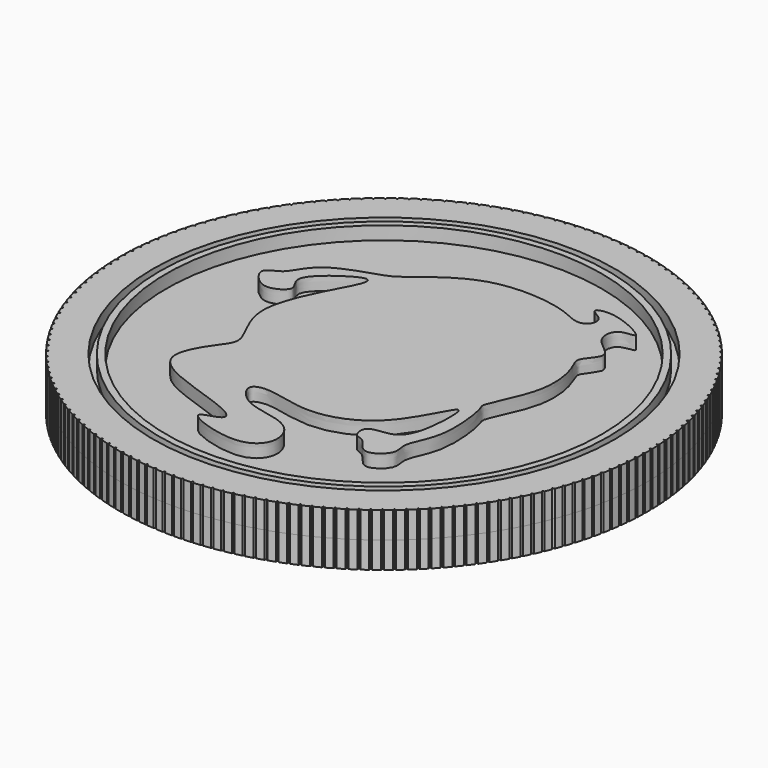
from build123d import *

# Parameters (mm, degrees)
F0_R     = 17.5
F0_R_2   = 17
F0_R_3   = 16.5
F2_DEPTH = 1
F3_DEPTH = 2
F4_DEPTH = 2


with BuildPart() as f2:
    # F0 (on Top) → F2 (new body)
    with BuildSketch(Plane.XY):
        with BuildLine():
            ThreePointArc((19.9982245618, -0.2664852267), (19.9995561355, -0.1332455705), (20, 0))
            ThreePointArc((20, 0), (19.9995561355, 0.1332455705), (19.9982245618, 0.2664852267))
            Line((19.9982245618, 0.2664852267), (19.8469084307, 0.3503223408))
            Line((19.8469084307, 0.3503223408), (19.9951715668, 0.4394473973))
            ThreePointArc((19.9951715668, 0.4394473973), (19.9875412452, 0.7058292781), (19.9763622593, 0.9720858433))
            Line((19.9763622593, 0.9720858433), (19.8221816542, 1.0505305643))
            Line((19.8221816542, 1.0505305643), (19.9672070779, 1.1448325245))
            ThreePointArc((19.9672070779, 1.1448325245), (19.950180503, 1.4107791808), (19.9296118969, 1.676475362))
            Line((19.9296118969, 1.676475362), (19.7727589077, 1.7494299575))
            Line((19.7727589077, 1.7494299575), (19.9143659353, 1.848791333))
            ThreePointArc((19.9143659353, 1.848791333), (19.8879643202, 2.1139714284), (19.8580317198, 2.3787762012))
            Line((19.8580317198, 2.3787762012), (19.6987017658, 2.4461497789))
            Line((19.6987017658, 2.4461497789), (19.8367139727, 2.5504467778))
            ThreePointArc((19.8367139727, 2.5504467778), (19.8009702103, 2.8145299308), (19.761710908, 3.0781133814))
            Line((19.761710908, 3.0781133814), (19.6001024945, 3.1398220023))
            Line((19.6001024945, 3.1398220023), (19.7343479345, 3.2489246834))
            ThreePointArc((19.7343479345, 3.2489246834), (19.6893065572, 3.5115818793), (19.6407694652, 3.7736156156))
            Line((19.6407694652, 3.7736156156), (19.4770839361, 3.8295823984))
            Line((19.4770839361, 3.8295823984), (19.6073953563, 3.9433548334))
            ThreePointArc((19.6073953563, 3.9433548334), (19.55311248, 4.2042588342), (19.4953580694, 4.4644163947))
            Line((19.4953580694, 4.4644163947), (19.3297993565, 4.5145716117))
            Line((19.3297993565, 4.5145716117), (19.456014405, 4.6328720544))
            ThreePointArc((19.456014405, 4.6328720544), (19.3925576594, 4.891697806), (19.3256578851, 5.1496550669))
            Line((19.3256578851, 5.1496550669), (19.1584322539, 5.193936231))
            Line((19.1584322539, 5.193936231), (19.2803936825, 5.3166172937))
            ThreePointArc((19.2803936825, 5.3166172937), (19.2078421269, 5.5730423315), (19.1318803376, 5.8284779101))
            Line((19.1318803376, 5.8284779101), (18.9631961305, 5.8668298525))
            Line((18.9631961305, 5.8668298525), (19.0807519904, 5.9937386899))
            ThreePointArc((19.0807519904, 5.9937386899), (18.9991960149, 6.2474435403), (18.9142668495, 6.5000391957))
            Line((18.9142668495, 6.5000391957), (18.744334226, 6.5324141345))
            Line((18.744334226, 6.5324141345), (18.8573380572, 6.663392634))
            ThreePointArc((18.8573380572, 6.663392634), (18.7668792705, 6.9140612123), (18.6730885402, 7.1635022418))
            Line((18.6730885402, 7.1635022418), (18.5021192152, 7.189859842))
            Line((18.5021192152, 7.189859842), (18.6104302291, 7.3247448207))
            ThreePointArc((18.6104302291, 7.3247448207), (18.5111813314, 7.5720648251), (18.4086458879, 7.8180404561))
            Line((18.4086458879, 7.8180404561), (18.2368528678, 7.8383478795))
            Line((18.2368528678, 7.8383478795), (18.3403361223, 7.9769712874))
            ThreePointArc((18.3403361223, 7.9769712874), (18.2324207655, 8.220634588), (18.1212683551, 8.4628383656))
            Line((18.1212683551, 8.4628383656), (17.9488656726, 8.4770703115))
            Line((17.9488656726, 8.4770703115), (18.0473922406, 8.6192594413))
            ThreePointArc((18.0473922406, 8.6192594413), (17.9309448737, 8.8589624638), (17.8113139785, 9.0970926323))
            Line((17.8113139785, 9.0970926323), (17.6385164259, 9.1052313695))
            Line((17.6385164259, 9.1052313695), (17.7319635554, 9.2508090711))
            ThreePointArc((17.7319635554, 9.2508090711), (17.6071292575, 9.4862531756), (17.4791689225, 9.7200130544))
            Line((17.4791689225, 9.7200130544), (17.3061917842, 9.7220484431))
            Line((17.3061917842, 9.7220484431), (17.3944430517, 9.8708333448))
            ThreePointArc((17.3944430517, 9.8708333448), (17.2613773506, 10.1017251972), (17.1252469987, 10.3308235506))
            Line((17.1252469987, 10.3308235506), (16.9523057825, 10.3267530549))
            Line((16.9523057825, 10.3267530549), (17.035251238, 10.4785597894))
            ThreePointArc((17.035251238, 10.4785597894), (16.8941199171, 10.704611727), (16.7499891496, 10.928763127))
            Line((16.7499891496, 10.928763127), (16.5772993188, 10.9185918184))
            Line((16.5772993188, 10.9185918184), (16.6548356225, 11.0732312532))
            ThreePointArc((16.6548356225, 11.0732312532), (16.5058145139, 11.2941616437), (16.3538628998, 11.5130868256))
            Line((16.3538628998, 11.5130868256), (16.1816396044, 11.4968273761))
            Line((16.1816396044, 11.4968273761), (16.2536701558, 11.6541068498))
            ThreePointArc((16.2536701558, 11.6541068498), (16.0969449211, 11.8696404413), (15.9373617733, 12.0830666516))
            Line((15.9373617733, 12.0830666516), (15.765819582, 12.0607393184))
            Line((15.765819582, 12.0607393184), (15.83225464, 12.2204628805))
            ThreePointArc((15.83225464, 12.2204628805), (15.6680205394, 12.4303311451), (15.5010046786, 12.6379924811))
            Line((15.5010046786, 12.6379924811), (15.3303573117, 12.6096250815))
            Line((15.3303573117, 12.6096250815), (15.3911141065, 12.7715937362))
            ThreePointArc((15.3911141065, 12.7715937362), (15.2195757552, 12.975535204), (15.0453352624, 13.1771729458))
            Line((15.0453352624, 13.1771729458), (14.8757953251, 13.1428008219))
            Line((14.8757953251, 13.1428008219), (14.9307981613, 13.3068127764))
            ThreePointArc((14.9307981613, 13.3068127764), (14.7521692748, 13.5045733619), (14.5709212318, 13.6999362938))
            Line((14.5709212318, 13.6999362938), (14.40269995, 13.6596022691))
            Line((14.40269995, 13.6596022691), (14.4518803009, 13.825453185))
            ThreePointArc((14.4518803009, 13.825453185), (14.2663834285, 14.016786503), (14.0783536479, 14.2056312272))
            Line((14.0783536479, 14.2056312272), (13.9116606043, 14.1593855528))
            Line((13.9116606043, 14.1593855528), (13.9549571972, 14.3268688004))
            ThreePointArc((13.9549571972, 14.3268688004), (13.7628234449, 14.5115364736), (13.5682461884, 14.6936277131))
            Line((13.5682461884, 14.6936277131), (13.4032890617, 14.6415280053))
            Line((13.4032890617, 14.6415280053), (13.4406479545, 14.8104349214))
            ThreePointArc((13.4406479545, 14.8104349214), (13.2421166971, 14.9882068767), (13.0412343837, 15.1633177685))
            Line((13.0412343837, 15.1633177685), (12.87821869, 15.1054289371))
            Line((12.87821869, 15.1054289371), (12.9095933382, 15.2755490848))
            ThreePointArc((12.9095933382, 15.2755490848), (12.7049119209, 15.4462038405), (12.497974825, 15.6141162182))
            Line((12.497974825, 15.6141162182), (12.3371036615, 15.5505103854))
            Line((12.3371036615, 15.5505103854), (12.3624549762, 15.7216318161))
            ThreePointArc((12.3624549762, 15.7216318161), (12.1518784065, 15.8849567577), (11.9391443459, 16.0454614234))
            Line((11.9391443459, 16.0454614234), (11.780618138, 15.9762178342))
            Line((11.780618138, 15.9762178342), (11.7999145347, 16.1481273519))
            ThreePointArc((11.7999145347, 16.1481273519), (11.5837051648, 16.3039189968), (11.3654391796, 16.4568159817))
            Line((11.3654391796, 16.4568159817), (11.2094554314, 16.382020905))
            Line((11.2094554314, 16.382020905), (11.222672869, 16.5545043319))
            ThreePointArc((11.222672869, 16.5545043319), (11.0011000689, 16.7025685831), (10.7775740914, 16.8476673965))
            Line((10.7775740914, 16.8476673965), (10.6243271391, 16.7674140177))
            Line((10.6243271391, 16.7674140177), (10.6314491505, 16.9402564609))
            ThreePointArc((10.6314491505, 16.9402564609), (10.4047889722, 17.0804088488), (10.176281488, 17.2175287157))
            Line((10.176281488, 17.2175287157), (10.0259622582, 17.1319170205))
            Line((10.0259622582, 17.1319170205), (10.0269799701, 17.3049031398))
            ThreePointArc((10.0269799701, 17.3049031398), (9.7955148041, 17.4369690521), (9.562310505, 17.5659391382))
            Line((9.562310505, 17.5659391382), (9.4151062768, 17.475075788))
            Line((9.4151062768, 17.475075788), (9.4100184214, 17.6479900643))
            ThreePointArc((9.4100184214, 17.6479900643), (9.1740366444, 17.7718049631), (8.9364260738, 17.8924645878))
            Line((8.9364260738, 17.8924645878), (8.7925202453, 17.7964627872))
            Line((8.7925202453, 17.7964627872), (8.7813331614, 17.9690897908))
            ThreePointArc((8.7813331614, 17.9690897908), (8.5411287773, 18.0844994183), (8.2994079686, 18.1966982546))
            Line((8.2994079686, 18.1966982546), (8.1589798285, 18.0956776098))
            Line((8.1589798285, 18.0956776098), (8.1417074538, 18.2678022689))
            ThreePointArc((8.1417074538, 18.2678022689), (7.8975797274, 18.3746628391), (7.6520498345, 18.4782611014))
            Line((7.6520498345, 18.4782611014), (7.5152743389, 18.3723474714))
            Line((7.5152743389, 18.3723474714), (7.4919381926, 18.5437553402))
            ThreePointArc((7.4919381926, 18.5437553402), (7.2441912766, 18.641933718), (6.9951581992, 18.7368023357))
            Line((6.9951581992, 18.7368023357), (6.8622057532, 18.6261276759))
            Line((6.8622057532, 18.6261276759), (6.8328349093, 18.7966052015))
            ThreePointArc((6.8328349093, 18.7966052015), (6.5817774655, 18.885979069), (6.3295514678, 18.9719998476))
            Line((6.3295514678, 18.9719998476), (6.2005877137, 18.8567020447))
            Line((6.2005877137, 18.8567020447), (6.1652187645, 19.0260368334))
            ThreePointArc((6.1652187645, 19.0260368334), (5.9111635793, 19.1064948418), (5.6560589035, 19.1835606101))
            Line((5.6560589035, 19.1835606101), (5.531244514, 19.0637833109))
            Line((5.531244514, 19.0637833109), (5.4899215249, 19.2317643925))
            ThreePointArc((5.4899215249, 19.2317643925), (5.2331851194, 19.3032063012), (4.9755195941, 19.3712210449))
            Line((4.9755195941, 19.3712210449), (4.8550100725, 19.247113477))
            Line((4.8550100725, 19.247113477), (4.8077845267, 19.4135315681))
            ThreePointArc((4.8077845267, 19.4135315681), (4.5486867624, 19.4758683693), (4.2887814069, 19.5347473504))
            Line((4.2887814069, 19.5347473504), (4.1727268929, 19.4064641364))
            Line((4.1727268929, 19.4064641364), (4.1196576277, 19.5711119007))
            ThreePointArc((4.1196576277, 19.5711119007), (3.8585213082, 19.6242659306), (3.5966999321, 19.6739357933))
            Line((3.5966999321, 19.6739357933), (3.4852450153, 19.5416367581))
            Line((3.4852450153, 19.5416367581), (3.4263981482, 19.704309065))
            ThreePointArc((3.4263981482, 19.704309065), (3.1635486169, 19.7482141002), (2.900137417, 19.7886129621))
            Line((2.900137417, 19.7886129621), (2.7934209563, 19.6524629337))
            Line((2.7934209563, 19.6524629337), (2.7288698034, 19.8129571139))
            ThreePointArc((2.7288698034, 19.8129571139), (2.4646345379, 19.8475584542), (2.1999616919, 19.8786359832))
            Line((2.1999616919, 19.8786359832), (2.0981166427, 19.7388045878))
            Line((2.0981166427, 19.7388045878), (2.0279416265, 19.8969206854))
            ThreePointArc((2.0279416265, 19.8969206854), (1.7626498313, 19.9221752219), (1.4970450884, 19.9438926994))
            Line((1.4970450884, 19.9438926994), (1.400198337, 19.8005541492))
            Line((1.400198337, 19.8005541492), (1.324486887, 19.9560951713))
            ThreePointArc((1.324486887, 19.9560951713), (1.0584690824, 19.97197144), (0.7922633532, 19.9843018086))
            Line((0.7922633532, 19.9843018086), (0.7005355585, 19.8376346859))
            Line((0.7005355585, 19.8376346859), (0.6193820017, 19.9904068477))
            ThreePointArc((0.6193820017, 19.9904068477), (0.3529696129, 19.9968850687), (0.0864945565, 19.9998129664))
            Line((0.0864945565, 19.9998129664), (0, 19.85))
            Line((0, 19.85), (-0.0864945565, 19.9998129664))
            ThreePointArc((-0.0864945565, 19.9998129664), (-0.3529696129, 19.9968850687), (-0.6193820017, 19.9904068477))
            Line((-0.6193820017, 19.9904068477), (-0.7005355585, 19.8376346859))
            Line((-0.7005355585, 19.8376346859), (-0.7922633532, 19.9843018086))
            ThreePointArc((-0.7922633532, 19.9843018086), (-1.0584690824, 19.97197144), (-1.324486887, 19.9560951713))
            Line((-1.324486887, 19.9560951713), (-1.400198337, 19.8005541492))
            Line((-1.400198337, 19.8005541492), (-1.4970450884, 19.9438926994))
            ThreePointArc((-1.4970450884, 19.9438926994), (-1.7626498313, 19.9221752219), (-2.0279416265, 19.8969206854))
            Line((-2.0279416265, 19.8969206854), (-2.0981166427, 19.7388045878))
            Line((-2.0981166427, 19.7388045878), (-2.1999616919, 19.8786359832))
            ThreePointArc((-2.1999616919, 19.8786359832), (-2.4646345379, 19.8475584542), (-2.7288698034, 19.8129571139))
            Line((-2.7288698034, 19.8129571139), (-2.7934209563, 19.6524629337))
            Line((-2.7934209563, 19.6524629337), (-2.900137417, 19.7886129621))
            ThreePointArc((-2.900137417, 19.7886129621), (-3.1635486169, 19.7482141002), (-3.4263981482, 19.704309065))
            Line((-3.4263981482, 19.704309065), (-3.4852450153, 19.5416367581))
            Line((-3.4852450153, 19.5416367581), (-3.5966999321, 19.6739357933))
            ThreePointArc((-3.5966999321, 19.6739357933), (-3.8585213082, 19.6242659306), (-4.1196576277, 19.5711119007))
            Line((-4.1196576277, 19.5711119007), (-4.1727268929, 19.4064641364))
            Line((-4.1727268929, 19.4064641364), (-4.2887814069, 19.5347473504))
            ThreePointArc((-4.2887814069, 19.5347473504), (-4.5486867624, 19.4758683693), (-4.8077845267, 19.4135315681))
            Line((-4.8077845267, 19.4135315681), (-4.8550100725, 19.247113477))
            Line((-4.8550100725, 19.247113477), (-4.9755195941, 19.3712210449))
            ThreePointArc((-4.9755195941, 19.3712210449), (-5.2331851194, 19.3032063012), (-5.4899215249, 19.2317643925))
            Line((-5.4899215249, 19.2317643925), (-5.531244514, 19.0637833109))
            Line((-5.531244514, 19.0637833109), (-5.6560589035, 19.1835606101))
            ThreePointArc((-5.6560589035, 19.1835606101), (-5.9111635793, 19.1064948418), (-6.1652187645, 19.0260368334))
            Line((-6.1652187645, 19.0260368334), (-6.2005877137, 18.8567020447))
            Line((-6.2005877137, 18.8567020447), (-6.3295514678, 18.9719998476))
            ThreePointArc((-6.3295514678, 18.9719998476), (-6.5817774655, 18.885979069), (-6.8328349093, 18.7966052015))
            Line((-6.8328349093, 18.7966052015), (-6.8622057532, 18.6261276759))
            Line((-6.8622057532, 18.6261276759), (-6.9951581992, 18.7368023357))
            ThreePointArc((-6.9951581992, 18.7368023357), (-7.2441912766, 18.641933718), (-7.4919381926, 18.5437553402))
            Line((-7.4919381926, 18.5437553402), (-7.5152743389, 18.3723474714))
            Line((-7.5152743389, 18.3723474714), (-7.6520498345, 18.4782611014))
            ThreePointArc((-7.6520498345, 18.4782611014), (-7.8975797274, 18.3746628391), (-8.1417074538, 18.2678022689))
            Line((-8.1417074538, 18.2678022689), (-8.1589798285, 18.0956776098))
            Line((-8.1589798285, 18.0956776098), (-8.2994079686, 18.1966982546))
            ThreePointArc((-8.2994079686, 18.1966982546), (-8.5411287773, 18.0844994183), (-8.7813331614, 17.9690897908))
            Line((-8.7813331614, 17.9690897908), (-8.7925202453, 17.7964627872))
            Line((-8.7925202453, 17.7964627872), (-8.9364260738, 17.8924645878))
            ThreePointArc((-8.9364260738, 17.8924645878), (-9.1740366444, 17.7718049631), (-9.4100184214, 17.6479900643))
            Line((-9.4100184214, 17.6479900643), (-9.4151062768, 17.475075788))
            Line((-9.4151062768, 17.475075788), (-9.562310505, 17.5659391382))
            ThreePointArc((-9.562310505, 17.5659391382), (-9.7955148041, 17.4369690521), (-10.0269799701, 17.3049031398))
            Line((-10.0269799701, 17.3049031398), (-10.0259622582, 17.1319170205))
            Line((-10.0259622582, 17.1319170205), (-10.176281488, 17.2175287157))
            ThreePointArc((-10.176281488, 17.2175287157), (-10.4047889722, 17.0804088488), (-10.6314491505, 16.9402564609))
            Line((-10.6314491505, 16.9402564609), (-10.6243271391, 16.7674140177))
            Line((-10.6243271391, 16.7674140177), (-10.7775740914, 16.8476673965))
            ThreePointArc((-10.7775740914, 16.8476673965), (-11.0011000689, 16.7025685831), (-11.222672869, 16.5545043319))
            Line((-11.222672869, 16.5545043319), (-11.2094554314, 16.382020905))
            Line((-11.2094554314, 16.382020905), (-11.3654391796, 16.4568159817))
            ThreePointArc((-11.3654391796, 16.4568159817), (-11.5837051648, 16.3039189968), (-11.7999145347, 16.1481273519))
            Line((-11.7999145347, 16.1481273519), (-11.780618138, 15.9762178342))
            Line((-11.780618138, 15.9762178342), (-11.9391443459, 16.0454614234))
            ThreePointArc((-11.9391443459, 16.0454614234), (-12.1518784065, 15.8849567577), (-12.3624549762, 15.7216318161))
            Line((-12.3624549762, 15.7216318161), (-12.3371036615, 15.5505103854))
            Line((-12.3371036615, 15.5505103854), (-12.497974825, 15.6141162182))
            ThreePointArc((-12.497974825, 15.6141162182), (-12.7049119209, 15.4462038405), (-12.9095933382, 15.2755490848))
            Line((-12.9095933382, 15.2755490848), (-12.87821869, 15.1054289371))
            Line((-12.87821869, 15.1054289371), (-13.0412343837, 15.1633177685))
            ThreePointArc((-13.0412343837, 15.1633177685), (-13.2421166971, 14.9882068767), (-13.4406479545, 14.8104349214))
            Line((-13.4406479545, 14.8104349214), (-13.4032890617, 14.6415280053))
            Line((-13.4032890617, 14.6415280053), (-13.5682461884, 14.6936277131))
            ThreePointArc((-13.5682461884, 14.6936277131), (-13.7628234449, 14.5115364736), (-13.9549571972, 14.3268688004))
            Line((-13.9549571972, 14.3268688004), (-13.9116606043, 14.1593855528))
            Line((-13.9116606043, 14.1593855528), (-14.0783536479, 14.2056312272))
            ThreePointArc((-14.0783536479, 14.2056312272), (-14.2663834285, 14.016786503), (-14.4518803009, 13.825453185))
            Line((-14.4518803009, 13.825453185), (-14.40269995, 13.6596022691))
            Line((-14.40269995, 13.6596022691), (-14.5709212318, 13.6999362938))
            ThreePointArc((-14.5709212318, 13.6999362938), (-14.7521692748, 13.5045733619), (-14.9307981613, 13.3068127764))
            Line((-14.9307981613, 13.3068127764), (-14.8757953251, 13.1428008219))
            Line((-14.8757953251, 13.1428008219), (-15.0453352624, 13.1771729458))
            ThreePointArc((-15.0453352624, 13.1771729458), (-15.2195757552, 12.975535204), (-15.3911141065, 12.7715937362))
            Line((-15.3911141065, 12.7715937362), (-15.3303573117, 12.6096250815))
            Line((-15.3303573117, 12.6096250815), (-15.5010046786, 12.6379924811))
            ThreePointArc((-15.5010046786, 12.6379924811), (-15.6680205394, 12.4303311451), (-15.83225464, 12.2204628805))
            Line((-15.83225464, 12.2204628805), (-15.765819582, 12.0607393184))
            Line((-15.765819582, 12.0607393184), (-15.9373617733, 12.0830666516))
            ThreePointArc((-15.9373617733, 12.0830666516), (-16.0969449211, 11.8696404413), (-16.2536701558, 11.6541068498))
            Line((-16.2536701558, 11.6541068498), (-16.1816396044, 11.4968273761))
            Line((-16.1816396044, 11.4968273761), (-16.3538628998, 11.5130868256))
            ThreePointArc((-16.3538628998, 11.5130868256), (-16.5058145139, 11.2941616437), (-16.6548356225, 11.0732312532))
            Line((-16.6548356225, 11.0732312532), (-16.5772993188, 10.9185918184))
            Line((-16.5772993188, 10.9185918184), (-16.7499891496, 10.928763127))
            ThreePointArc((-16.7499891496, 10.928763127), (-16.8941199171, 10.704611727), (-17.035251238, 10.4785597894))
            Line((-17.035251238, 10.4785597894), (-16.9523057825, 10.3267530549))
            Line((-16.9523057825, 10.3267530549), (-17.1252469987, 10.3308235506))
            ThreePointArc((-17.1252469987, 10.3308235506), (-17.2613773506, 10.1017251972), (-17.3944430517, 9.8708333448))
            Line((-17.3944430517, 9.8708333448), (-17.3061917842, 9.7220484431))
            Line((-17.3061917842, 9.7220484431), (-17.4791689225, 9.7200130544))
            ThreePointArc((-17.4791689225, 9.7200130544), (-17.6071292575, 9.4862531756), (-17.7319635554, 9.2508090711))
            Line((-17.7319635554, 9.2508090711), (-17.6385164259, 9.1052313695))
            Line((-17.6385164259, 9.1052313695), (-17.8113139785, 9.0970926323))
            ThreePointArc((-17.8113139785, 9.0970926323), (-17.9309448737, 8.8589624638), (-18.0473922406, 8.6192594413))
            Line((-18.0473922406, 8.6192594413), (-17.9488656726, 8.4770703115))
            Line((-17.9488656726, 8.4770703115), (-18.1212683551, 8.4628383656))
            ThreePointArc((-18.1212683551, 8.4628383656), (-18.2324207655, 8.220634588), (-18.3403361223, 7.9769712874))
            Line((-18.3403361223, 7.9769712874), (-18.2368528678, 7.8383478795))
            Line((-18.2368528678, 7.8383478795), (-18.4086458879, 7.8180404561))
            ThreePointArc((-18.4086458879, 7.8180404561), (-18.5111813314, 7.5720648251), (-18.6104302291, 7.3247448207))
            Line((-18.6104302291, 7.3247448207), (-18.5021192152, 7.189859842))
            Line((-18.5021192152, 7.189859842), (-18.6730885402, 7.1635022418))
            ThreePointArc((-18.6730885402, 7.1635022418), (-18.7668792705, 6.9140612123), (-18.8573380572, 6.663392634))
            Line((-18.8573380572, 6.663392634), (-18.744334226, 6.5324141345))
            Line((-18.744334226, 6.5324141345), (-18.9142668495, 6.5000391957))
            ThreePointArc((-18.9142668495, 6.5000391957), (-18.9991960149, 6.2474435403), (-19.0807519904, 5.9937386899))
            Line((-19.0807519904, 5.9937386899), (-18.9631961305, 5.8668298525))
            Line((-18.9631961305, 5.8668298525), (-19.1318803376, 5.8284779101))
            ThreePointArc((-19.1318803376, 5.8284779101), (-19.2078421269, 5.5730423315), (-19.2803936825, 5.3166172937))
            Line((-19.2803936825, 5.3166172937), (-19.1584322539, 5.193936231))
            Line((-19.1584322539, 5.193936231), (-19.3256578851, 5.1496550669))
            ThreePointArc((-19.3256578851, 5.1496550669), (-19.3925576594, 4.891697806), (-19.456014405, 4.6328720544))
            Line((-19.456014405, 4.6328720544), (-19.3297993565, 4.5145716117))
            Line((-19.3297993565, 4.5145716117), (-19.4953580694, 4.4644163947))
            ThreePointArc((-19.4953580694, 4.4644163947), (-19.55311248, 4.2042588342), (-19.6073953563, 3.9433548334))
            Line((-19.6073953563, 3.9433548334), (-19.4770839361, 3.8295823984))
            Line((-19.4770839361, 3.8295823984), (-19.6407694652, 3.7736156156))
            ThreePointArc((-19.6407694652, 3.7736156156), (-19.6893065572, 3.5115818793), (-19.7343479345, 3.2489246834))
            Line((-19.7343479345, 3.2489246834), (-19.6001024945, 3.1398220023))
            Line((-19.6001024945, 3.1398220023), (-19.761710908, 3.0781133814))
            ThreePointArc((-19.761710908, 3.0781133814), (-19.8009702103, 2.8145299308), (-19.8367139727, 2.5504467778))
            Line((-19.8367139727, 2.5504467778), (-19.6987017658, 2.4461497789))
            Line((-19.6987017658, 2.4461497789), (-19.8580317198, 2.3787762012))
            ThreePointArc((-19.8580317198, 2.3787762012), (-19.8879643202, 2.1139714284), (-19.9143659353, 1.848791333))
            Line((-19.9143659353, 1.848791333), (-19.7727589077, 1.7494299575))
            Line((-19.7727589077, 1.7494299575), (-19.9296118969, 1.676475362))
            ThreePointArc((-19.9296118969, 1.676475362), (-19.950180503, 1.4107791808), (-19.9672070779, 1.1448325245))
            Line((-19.9672070779, 1.1448325245), (-19.8221816542, 1.0505305643))
            Line((-19.8221816542, 1.0505305643), (-19.9763622593, 0.9720858433))
            ThreePointArc((-19.9763622593, 0.9720858433), (-19.9875412452, 0.7058292781), (-19.9951715668, 0.4394473973))
            Line((-19.9951715668, 0.4394473973), (-19.8469084307, 0.3503223408))
            Line((-19.8469084307, 0.3503223408), (-19.9982245618, 0.2664852267))
            ThreePointArc((-19.9982245618, 0.2664852267), (-20, 0), (-19.9982245618, -0.2664852267))
            Line((-19.9982245618, -0.2664852267), (-19.8469084307, -0.3503223408))
            Line((-19.8469084307, -0.3503223408), (-19.9951715668, -0.4394473973))
            ThreePointArc((-19.9951715668, -0.4394473973), (-19.9875412452, -0.7058292781), (-19.9763622593, -0.9720858433))
            Line((-19.9763622593, -0.9720858433), (-19.8221816542, -1.0505305643))
            Line((-19.8221816542, -1.0505305643), (-19.9672070779, -1.1448325245))
            ThreePointArc((-19.9672070779, -1.1448325245), (-19.950180503, -1.4107791808), (-19.9296118969, -1.676475362))
            Line((-19.9296118969, -1.676475362), (-19.7727589077, -1.7494299575))
            Line((-19.7727589077, -1.7494299575), (-19.9143659353, -1.848791333))
            ThreePointArc((-19.9143659353, -1.848791333), (-19.8879643202, -2.1139714284), (-19.8580317198, -2.3787762012))
            Line((-19.8580317198, -2.3787762012), (-19.6987017658, -2.4461497789))
            Line((-19.6987017658, -2.4461497789), (-19.8367139727, -2.5504467778))
            ThreePointArc((-19.8367139727, -2.5504467778), (-19.8009702103, -2.8145299308), (-19.761710908, -3.0781133814))
            Line((-19.761710908, -3.0781133814), (-19.6001024945, -3.1398220023))
            Line((-19.6001024945, -3.1398220023), (-19.7343479345, -3.2489246834))
            ThreePointArc((-19.7343479345, -3.2489246834), (-19.6893065572, -3.5115818793), (-19.6407694652, -3.7736156156))
            Line((-19.6407694652, -3.7736156156), (-19.4770839361, -3.8295823984))
            Line((-19.4770839361, -3.8295823984), (-19.6073953563, -3.9433548334))
            ThreePointArc((-19.6073953563, -3.9433548334), (-19.55311248, -4.2042588342), (-19.4953580694, -4.4644163947))
            Line((-19.4953580694, -4.4644163947), (-19.3297993565, -4.5145716117))
            Line((-19.3297993565, -4.5145716117), (-19.456014405, -4.6328720544))
            ThreePointArc((-19.456014405, -4.6328720544), (-19.3925576594, -4.891697806), (-19.3256578851, -5.1496550669))
            Line((-19.3256578851, -5.1496550669), (-19.1584322539, -5.193936231))
            Line((-19.1584322539, -5.193936231), (-19.2803936825, -5.3166172937))
            ThreePointArc((-19.2803936825, -5.3166172937), (-19.2078421269, -5.5730423315), (-19.1318803376, -5.8284779101))
            Line((-19.1318803376, -5.8284779101), (-18.9631961305, -5.8668298525))
            Line((-18.9631961305, -5.8668298525), (-19.0807519904, -5.9937386899))
            ThreePointArc((-19.0807519904, -5.9937386899), (-18.9991960149, -6.2474435403), (-18.9142668495, -6.5000391957))
            Line((-18.9142668495, -6.5000391957), (-18.744334226, -6.5324141345))
            Line((-18.744334226, -6.5324141345), (-18.8573380572, -6.663392634))
            ThreePointArc((-18.8573380572, -6.663392634), (-18.7668792705, -6.9140612123), (-18.6730885402, -7.1635022418))
            Line((-18.6730885402, -7.1635022418), (-18.5021192152, -7.189859842))
            Line((-18.5021192152, -7.189859842), (-18.6104302291, -7.3247448207))
            ThreePointArc((-18.6104302291, -7.3247448207), (-18.5111813314, -7.5720648251), (-18.4086458879, -7.8180404561))
            Line((-18.4086458879, -7.8180404561), (-18.2368528678, -7.8383478795))
            Line((-18.2368528678, -7.8383478795), (-18.3403361223, -7.9769712874))
            ThreePointArc((-18.3403361223, -7.9769712874), (-18.2324207655, -8.220634588), (-18.1212683551, -8.4628383656))
            Line((-18.1212683551, -8.4628383656), (-17.9488656726, -8.4770703115))
            Line((-17.9488656726, -8.4770703115), (-18.0473922406, -8.6192594413))
            ThreePointArc((-18.0473922406, -8.6192594413), (-17.9309448737, -8.8589624638), (-17.8113139785, -9.0970926323))
            Line((-17.8113139785, -9.0970926323), (-17.6385164259, -9.1052313695))
            Line((-17.6385164259, -9.1052313695), (-17.7319635554, -9.2508090711))
            ThreePointArc((-17.7319635554, -9.2508090711), (-17.6071292575, -9.4862531756), (-17.4791689225, -9.7200130544))
            Line((-17.4791689225, -9.7200130544), (-17.3061917842, -9.7220484431))
            Line((-17.3061917842, -9.7220484431), (-17.3944430517, -9.8708333448))
            ThreePointArc((-17.3944430517, -9.8708333448), (-17.2613773506, -10.1017251972), (-17.1252469987, -10.3308235506))
            Line((-17.1252469987, -10.3308235506), (-16.9523057825, -10.3267530549))
            Line((-16.9523057825, -10.3267530549), (-17.035251238, -10.4785597894))
            ThreePointArc((-17.035251238, -10.4785597894), (-16.8941199171, -10.704611727), (-16.7499891496, -10.928763127))
            Line((-16.7499891496, -10.928763127), (-16.5772993188, -10.9185918184))
            Line((-16.5772993188, -10.9185918184), (-16.6548356225, -11.0732312532))
            ThreePointArc((-16.6548356225, -11.0732312532), (-16.5058145139, -11.2941616437), (-16.3538628998, -11.5130868256))
            Line((-16.3538628998, -11.5130868256), (-16.1816396044, -11.4968273761))
            Line((-16.1816396044, -11.4968273761), (-16.2536701558, -11.6541068498))
            ThreePointArc((-16.2536701558, -11.6541068498), (-16.0969449211, -11.8696404413), (-15.9373617733, -12.0830666516))
            Line((-15.9373617733, -12.0830666516), (-15.765819582, -12.0607393184))
            Line((-15.765819582, -12.0607393184), (-15.83225464, -12.2204628805))
            ThreePointArc((-15.83225464, -12.2204628805), (-15.6680205394, -12.4303311451), (-15.5010046786, -12.6379924811))
            Line((-15.5010046786, -12.6379924811), (-15.3303573117, -12.6096250815))
            Line((-15.3303573117, -12.6096250815), (-15.3911141065, -12.7715937362))
            ThreePointArc((-15.3911141065, -12.7715937362), (-15.2195757552, -12.975535204), (-15.0453352624, -13.1771729458))
            Line((-15.0453352624, -13.1771729458), (-14.8757953251, -13.1428008219))
            Line((-14.8757953251, -13.1428008219), (-14.9307981613, -13.3068127764))
            ThreePointArc((-14.9307981613, -13.3068127764), (-14.7521692748, -13.5045733619), (-14.5709212318, -13.6999362938))
            Line((-14.5709212318, -13.6999362938), (-14.40269995, -13.6596022691))
            Line((-14.40269995, -13.6596022691), (-14.4518803009, -13.825453185))
            ThreePointArc((-14.4518803009, -13.825453185), (-14.2663834285, -14.016786503), (-14.0783536479, -14.2056312272))
            Line((-14.0783536479, -14.2056312272), (-13.9116606043, -14.1593855528))
            Line((-13.9116606043, -14.1593855528), (-13.9549571972, -14.3268688004))
            ThreePointArc((-13.9549571972, -14.3268688004), (-13.7628234449, -14.5115364736), (-13.5682461884, -14.6936277131))
            Line((-13.5682461884, -14.6936277131), (-13.4032890617, -14.6415280053))
            Line((-13.4032890617, -14.6415280053), (-13.4406479545, -14.8104349214))
            ThreePointArc((-13.4406479545, -14.8104349214), (-13.2421166971, -14.9882068767), (-13.0412343837, -15.1633177685))
            Line((-13.0412343837, -15.1633177685), (-12.87821869, -15.1054289371))
            Line((-12.87821869, -15.1054289371), (-12.9095933382, -15.2755490848))
            ThreePointArc((-12.9095933382, -15.2755490848), (-12.7049119209, -15.4462038405), (-12.497974825, -15.6141162182))
            Line((-12.497974825, -15.6141162182), (-12.3371036615, -15.5505103854))
            Line((-12.3371036615, -15.5505103854), (-12.3624549762, -15.7216318161))
            ThreePointArc((-12.3624549762, -15.7216318161), (-12.1518784065, -15.8849567577), (-11.9391443459, -16.0454614234))
            Line((-11.9391443459, -16.0454614234), (-11.780618138, -15.9762178342))
            Line((-11.780618138, -15.9762178342), (-11.7999145347, -16.1481273519))
            ThreePointArc((-11.7999145347, -16.1481273519), (-11.5837051648, -16.3039189968), (-11.3654391796, -16.4568159817))
            Line((-11.3654391796, -16.4568159817), (-11.2094554314, -16.382020905))
            Line((-11.2094554314, -16.382020905), (-11.222672869, -16.5545043319))
            ThreePointArc((-11.222672869, -16.5545043319), (-11.0011000689, -16.7025685831), (-10.7775740914, -16.8476673965))
            Line((-10.7775740914, -16.8476673965), (-10.6243271391, -16.7674140177))
            Line((-10.6243271391, -16.7674140177), (-10.6314491505, -16.9402564609))
            ThreePointArc((-10.6314491505, -16.9402564609), (-10.4047889722, -17.0804088488), (-10.176281488, -17.2175287157))
            Line((-10.176281488, -17.2175287157), (-10.0259622582, -17.1319170205))
            Line((-10.0259622582, -17.1319170205), (-10.0269799701, -17.3049031398))
            ThreePointArc((-10.0269799701, -17.3049031398), (-9.7955148041, -17.4369690521), (-9.562310505, -17.5659391382))
            Line((-9.562310505, -17.5659391382), (-9.4151062768, -17.475075788))
            Line((-9.4151062768, -17.475075788), (-9.4100184214, -17.6479900643))
            ThreePointArc((-9.4100184214, -17.6479900643), (-9.1740366444, -17.7718049631), (-8.9364260738, -17.8924645878))
            Line((-8.9364260738, -17.8924645878), (-8.7925202453, -17.7964627872))
            Line((-8.7925202453, -17.7964627872), (-8.7813331614, -17.9690897908))
            ThreePointArc((-8.7813331614, -17.9690897908), (-8.5411287773, -18.0844994183), (-8.2994079686, -18.1966982546))
            Line((-8.2994079686, -18.1966982546), (-8.1589798285, -18.0956776098))
            Line((-8.1589798285, -18.0956776098), (-8.1417074538, -18.2678022689))
            ThreePointArc((-8.1417074538, -18.2678022689), (-7.8975797274, -18.3746628391), (-7.6520498345, -18.4782611014))
            Line((-7.6520498345, -18.4782611014), (-7.5152743389, -18.3723474714))
            Line((-7.5152743389, -18.3723474714), (-7.4919381926, -18.5437553402))
            ThreePointArc((-7.4919381926, -18.5437553402), (-7.2441912766, -18.641933718), (-6.9951581992, -18.7368023357))
            Line((-6.9951581992, -18.7368023357), (-6.8622057532, -18.6261276759))
            Line((-6.8622057532, -18.6261276759), (-6.8328349093, -18.7966052015))
            ThreePointArc((-6.8328349093, -18.7966052015), (-6.5817774655, -18.885979069), (-6.3295514678, -18.9719998476))
            Line((-6.3295514678, -18.9719998476), (-6.2005877137, -18.8567020447))
            Line((-6.2005877137, -18.8567020447), (-6.1652187645, -19.0260368334))
            ThreePointArc((-6.1652187645, -19.0260368334), (-5.9111635793, -19.1064948418), (-5.6560589035, -19.1835606101))
            Line((-5.6560589035, -19.1835606101), (-5.531244514, -19.0637833109))
            Line((-5.531244514, -19.0637833109), (-5.4899215249, -19.2317643925))
            ThreePointArc((-5.4899215249, -19.2317643925), (-5.2331851194, -19.3032063012), (-4.9755195941, -19.3712210449))
            Line((-4.9755195941, -19.3712210449), (-4.8550100725, -19.247113477))
            Line((-4.8550100725, -19.247113477), (-4.8077845267, -19.4135315681))
            ThreePointArc((-4.8077845267, -19.4135315681), (-4.5486867624, -19.4758683693), (-4.2887814069, -19.5347473504))
            Line((-4.2887814069, -19.5347473504), (-4.1727268929, -19.4064641364))
            Line((-4.1727268929, -19.4064641364), (-4.1196576277, -19.5711119007))
            ThreePointArc((-4.1196576277, -19.5711119007), (-3.8585213082, -19.6242659306), (-3.5966999321, -19.6739357933))
            Line((-3.5966999321, -19.6739357933), (-3.4852450153, -19.5416367581))
            Line((-3.4852450153, -19.5416367581), (-3.4263981482, -19.704309065))
            ThreePointArc((-3.4263981482, -19.704309065), (-3.1635486169, -19.7482141002), (-2.900137417, -19.7886129621))
            Line((-2.900137417, -19.7886129621), (-2.7934209563, -19.6524629337))
            Line((-2.7934209563, -19.6524629337), (-2.7288698034, -19.8129571139))
            ThreePointArc((-2.7288698034, -19.8129571139), (-2.4646345379, -19.8475584542), (-2.1999616919, -19.8786359832))
            Line((-2.1999616919, -19.8786359832), (-2.0981166427, -19.7388045878))
            Line((-2.0981166427, -19.7388045878), (-2.0279416265, -19.8969206854))
            ThreePointArc((-2.0279416265, -19.8969206854), (-1.7626498313, -19.9221752219), (-1.4970450884, -19.9438926994))
            Line((-1.4970450884, -19.9438926994), (-1.400198337, -19.8005541492))
            Line((-1.400198337, -19.8005541492), (-1.324486887, -19.9560951713))
            ThreePointArc((-1.324486887, -19.9560951713), (-1.0584690824, -19.97197144), (-0.7922633532, -19.9843018086))
            Line((-0.7922633532, -19.9843018086), (-0.7005355585, -19.8376346859))
            Line((-0.7005355585, -19.8376346859), (-0.6193820017, -19.9904068477))
            ThreePointArc((-0.6193820017, -19.9904068477), (-0.3529696129, -19.9968850687), (-0.0864945565, -19.9998129664))
            Line((-0.0864945565, -19.9998129664), (0, -19.85))
            Line((0, -19.85), (0.0864945565, -19.9998129664))
            ThreePointArc((0.0864945565, -19.9998129664), (0.3529696129, -19.9968850687), (0.6193820017, -19.9904068477))
            Line((0.6193820017, -19.9904068477), (0.7005355585, -19.8376346859))
            Line((0.7005355585, -19.8376346859), (0.7922633532, -19.9843018086))
            ThreePointArc((0.7922633532, -19.9843018086), (1.0584690824, -19.97197144), (1.324486887, -19.9560951713))
            Line((1.324486887, -19.9560951713), (1.400198337, -19.8005541492))
            Line((1.400198337, -19.8005541492), (1.4970450884, -19.9438926994))
            ThreePointArc((1.4970450884, -19.9438926994), (1.7626498313, -19.9221752219), (2.0279416265, -19.8969206854))
            Line((2.0279416265, -19.8969206854), (2.0981166427, -19.7388045878))
            Line((2.0981166427, -19.7388045878), (2.1999616919, -19.8786359832))
            ThreePointArc((2.1999616919, -19.8786359832), (2.4646345379, -19.8475584542), (2.7288698034, -19.8129571139))
            Line((2.7288698034, -19.8129571139), (2.7934209563, -19.6524629337))
            Line((2.7934209563, -19.6524629337), (2.900137417, -19.7886129621))
            ThreePointArc((2.900137417, -19.7886129621), (3.1635486169, -19.7482141002), (3.4263981482, -19.704309065))
            Line((3.4263981482, -19.704309065), (3.4852450153, -19.5416367581))
            Line((3.4852450153, -19.5416367581), (3.5966999321, -19.6739357933))
            ThreePointArc((3.5966999321, -19.6739357933), (3.8585213082, -19.6242659306), (4.1196576277, -19.5711119007))
            Line((4.1196576277, -19.5711119007), (4.1727268929, -19.4064641364))
            Line((4.1727268929, -19.4064641364), (4.2887814069, -19.5347473504))
            ThreePointArc((4.2887814069, -19.5347473504), (4.5486867624, -19.4758683693), (4.8077845267, -19.4135315681))
            Line((4.8077845267, -19.4135315681), (4.8550100725, -19.247113477))
            Line((4.8550100725, -19.247113477), (4.9755195941, -19.3712210449))
            ThreePointArc((4.9755195941, -19.3712210449), (5.2331851194, -19.3032063012), (5.4899215249, -19.2317643925))
            Line((5.4899215249, -19.2317643925), (5.531244514, -19.0637833109))
            Line((5.531244514, -19.0637833109), (5.6560589035, -19.1835606101))
            ThreePointArc((5.6560589035, -19.1835606101), (5.9111635793, -19.1064948418), (6.1652187645, -19.0260368334))
            Line((6.1652187645, -19.0260368334), (6.2005877137, -18.8567020447))
            Line((6.2005877137, -18.8567020447), (6.3295514678, -18.9719998476))
            ThreePointArc((6.3295514678, -18.9719998476), (6.5817774655, -18.885979069), (6.8328349093, -18.7966052015))
            Line((6.8328349093, -18.7966052015), (6.8622057532, -18.6261276759))
            Line((6.8622057532, -18.6261276759), (6.9951581992, -18.7368023357))
            ThreePointArc((6.9951581992, -18.7368023357), (7.2441912766, -18.641933718), (7.4919381926, -18.5437553402))
            Line((7.4919381926, -18.5437553402), (7.5152743389, -18.3723474714))
            Line((7.5152743389, -18.3723474714), (7.6520498345, -18.4782611014))
            ThreePointArc((7.6520498345, -18.4782611014), (7.8975797274, -18.3746628391), (8.1417074538, -18.2678022689))
            Line((8.1417074538, -18.2678022689), (8.1589798285, -18.0956776098))
            Line((8.1589798285, -18.0956776098), (8.2994079686, -18.1966982546))
            ThreePointArc((8.2994079686, -18.1966982546), (8.5411287773, -18.0844994183), (8.7813331614, -17.9690897908))
            Line((8.7813331614, -17.9690897908), (8.7925202453, -17.7964627872))
            Line((8.7925202453, -17.7964627872), (8.9364260738, -17.8924645878))
            ThreePointArc((8.9364260738, -17.8924645878), (9.1740366444, -17.7718049631), (9.4100184214, -17.6479900643))
            Line((9.4100184214, -17.6479900643), (9.4151062768, -17.475075788))
            Line((9.4151062768, -17.475075788), (9.562310505, -17.5659391382))
            ThreePointArc((9.562310505, -17.5659391382), (9.7955148041, -17.4369690521), (10.0269799701, -17.3049031398))
            Line((10.0269799701, -17.3049031398), (10.0259622582, -17.1319170205))
            Line((10.0259622582, -17.1319170205), (10.176281488, -17.2175287157))
            ThreePointArc((10.176281488, -17.2175287157), (10.4047889722, -17.0804088488), (10.6314491505, -16.9402564609))
            Line((10.6314491505, -16.9402564609), (10.6243271391, -16.7674140177))
            Line((10.6243271391, -16.7674140177), (10.7775740914, -16.8476673965))
            ThreePointArc((10.7775740914, -16.8476673965), (11.0011000689, -16.7025685831), (11.222672869, -16.5545043319))
            Line((11.222672869, -16.5545043319), (11.2094554314, -16.382020905))
            Line((11.2094554314, -16.382020905), (11.3654391796, -16.4568159817))
            ThreePointArc((11.3654391796, -16.4568159817), (11.5837051648, -16.3039189968), (11.7999145347, -16.1481273519))
            Line((11.7999145347, -16.1481273519), (11.780618138, -15.9762178342))
            Line((11.780618138, -15.9762178342), (11.9391443459, -16.0454614234))
            ThreePointArc((11.9391443459, -16.0454614234), (12.1518784065, -15.8849567577), (12.3624549762, -15.7216318161))
            Line((12.3624549762, -15.7216318161), (12.3371036615, -15.5505103854))
            Line((12.3371036615, -15.5505103854), (12.497974825, -15.6141162182))
            ThreePointArc((12.497974825, -15.6141162182), (12.7049119209, -15.4462038405), (12.9095933382, -15.2755490848))
            Line((12.9095933382, -15.2755490848), (12.87821869, -15.1054289371))
            Line((12.87821869, -15.1054289371), (13.0412343837, -15.1633177685))
            ThreePointArc((13.0412343837, -15.1633177685), (13.2421166971, -14.9882068767), (13.4406479545, -14.8104349214))
            Line((13.4406479545, -14.8104349214), (13.4032890617, -14.6415280053))
            Line((13.4032890617, -14.6415280053), (13.5682461884, -14.6936277131))
            ThreePointArc((13.5682461884, -14.6936277131), (13.7628234449, -14.5115364736), (13.9549571972, -14.3268688004))
            Line((13.9549571972, -14.3268688004), (13.9116606043, -14.1593855528))
            Line((13.9116606043, -14.1593855528), (14.0783536479, -14.2056312272))
            ThreePointArc((14.0783536479, -14.2056312272), (14.2663834285, -14.016786503), (14.4518803009, -13.825453185))
            Line((14.4518803009, -13.825453185), (14.40269995, -13.6596022691))
            Line((14.40269995, -13.6596022691), (14.5709212318, -13.6999362938))
            ThreePointArc((14.5709212318, -13.6999362938), (14.7521692748, -13.5045733619), (14.9307981613, -13.3068127764))
            Line((14.9307981613, -13.3068127764), (14.8757953251, -13.1428008219))
            Line((14.8757953251, -13.1428008219), (15.0453352624, -13.1771729458))
            ThreePointArc((15.0453352624, -13.1771729458), (15.2195757552, -12.975535204), (15.3911141065, -12.7715937362))
            Line((15.3911141065, -12.7715937362), (15.3303573117, -12.6096250815))
            Line((15.3303573117, -12.6096250815), (15.5010046786, -12.6379924811))
            ThreePointArc((15.5010046786, -12.6379924811), (15.6680205394, -12.4303311451), (15.83225464, -12.2204628805))
            Line((15.83225464, -12.2204628805), (15.765819582, -12.0607393184))
            Line((15.765819582, -12.0607393184), (15.9373617733, -12.0830666516))
            ThreePointArc((15.9373617733, -12.0830666516), (16.0969449211, -11.8696404413), (16.2536701558, -11.6541068498))
            Line((16.2536701558, -11.6541068498), (16.1816396044, -11.4968273761))
            Line((16.1816396044, -11.4968273761), (16.3538628998, -11.5130868256))
            ThreePointArc((16.3538628998, -11.5130868256), (16.5058145139, -11.2941616437), (16.6548356225, -11.0732312532))
            Line((16.6548356225, -11.0732312532), (16.5772993188, -10.9185918184))
            Line((16.5772993188, -10.9185918184), (16.7499891496, -10.928763127))
            ThreePointArc((16.7499891496, -10.928763127), (16.8941199171, -10.704611727), (17.035251238, -10.4785597894))
            Line((17.035251238, -10.4785597894), (16.9523057825, -10.3267530549))
            Line((16.9523057825, -10.3267530549), (17.1252469987, -10.3308235506))
            ThreePointArc((17.1252469987, -10.3308235506), (17.2613773506, -10.1017251972), (17.3944430517, -9.8708333448))
            Line((17.3944430517, -9.8708333448), (17.3061917842, -9.7220484431))
            Line((17.3061917842, -9.7220484431), (17.4791689225, -9.7200130544))
            ThreePointArc((17.4791689225, -9.7200130544), (17.6071292575, -9.4862531756), (17.7319635554, -9.2508090711))
            Line((17.7319635554, -9.2508090711), (17.6385164259, -9.1052313695))
            Line((17.6385164259, -9.1052313695), (17.8113139785, -9.0970926323))
            ThreePointArc((17.8113139785, -9.0970926323), (17.9309448737, -8.8589624638), (18.0473922406, -8.6192594413))
            Line((18.0473922406, -8.6192594413), (17.9488656726, -8.4770703115))
            Line((17.9488656726, -8.4770703115), (18.1212683551, -8.4628383656))
            ThreePointArc((18.1212683551, -8.4628383656), (18.2324207655, -8.220634588), (18.3403361223, -7.9769712874))
            Line((18.3403361223, -7.9769712874), (18.2368528678, -7.8383478795))
            Line((18.2368528678, -7.8383478795), (18.4086458879, -7.8180404561))
            ThreePointArc((18.4086458879, -7.8180404561), (18.5111813314, -7.5720648251), (18.6104302291, -7.3247448207))
            Line((18.6104302291, -7.3247448207), (18.5021192152, -7.189859842))
            Line((18.5021192152, -7.189859842), (18.6730885402, -7.1635022418))
            ThreePointArc((18.6730885402, -7.1635022418), (18.7668792705, -6.9140612123), (18.8573380572, -6.663392634))
            Line((18.8573380572, -6.663392634), (18.744334226, -6.5324141345))
            Line((18.744334226, -6.5324141345), (18.9142668495, -6.5000391957))
            ThreePointArc((18.9142668495, -6.5000391957), (18.9991960149, -6.2474435403), (19.0807519904, -5.9937386899))
            Line((19.0807519904, -5.9937386899), (18.9631961305, -5.8668298525))
            Line((18.9631961305, -5.8668298525), (19.1318803376, -5.8284779101))
            ThreePointArc((19.1318803376, -5.8284779101), (19.2078421269, -5.5730423315), (19.2803936825, -5.3166172937))
            Line((19.2803936825, -5.3166172937), (19.1584322539, -5.193936231))
            Line((19.1584322539, -5.193936231), (19.3256578851, -5.1496550669))
            ThreePointArc((19.3256578851, -5.1496550669), (19.3925576594, -4.891697806), (19.456014405, -4.6328720544))
            Line((19.456014405, -4.6328720544), (19.3297993565, -4.5145716117))
            Line((19.3297993565, -4.5145716117), (19.4953580694, -4.4644163947))
            ThreePointArc((19.4953580694, -4.4644163947), (19.55311248, -4.2042588342), (19.6073953563, -3.9433548334))
            Line((19.6073953563, -3.9433548334), (19.4770839361, -3.8295823984))
            Line((19.4770839361, -3.8295823984), (19.6407694652, -3.7736156156))
            ThreePointArc((19.6407694652, -3.7736156156), (19.6893065572, -3.5115818793), (19.7343479345, -3.2489246834))
            Line((19.7343479345, -3.2489246834), (19.6001024945, -3.1398220023))
            Line((19.6001024945, -3.1398220023), (19.761710908, -3.0781133814))
            ThreePointArc((19.761710908, -3.0781133814), (19.8009702103, -2.8145299308), (19.8367139727, -2.5504467778))
            Line((19.8367139727, -2.5504467778), (19.6987017658, -2.4461497789))
            Line((19.6987017658, -2.4461497789), (19.8580317198, -2.3787762012))
            ThreePointArc((19.8580317198, -2.3787762012), (19.8879643202, -2.1139714284), (19.9143659353, -1.848791333))
            Line((19.9143659353, -1.848791333), (19.7727589077, -1.7494299575))
            Line((19.7727589077, -1.7494299575), (19.9296118969, -1.676475362))
            ThreePointArc((19.9296118969, -1.676475362), (19.950180503, -1.4107791808), (19.9672070779, -1.1448325245))
            Line((19.9672070779, -1.1448325245), (19.8221816542, -1.0505305643))
            Line((19.8221816542, -1.0505305643), (19.9763622593, -0.9720858433))
            ThreePointArc((19.9763622593, -0.9720858433), (19.9875412452, -0.7058292781), (19.9951715668, -0.4394473973))
            Line((19.9951715668, -0.4394473973), (19.8469084307, -0.3503223408))
            Line((19.8469084307, -0.3503223408), (19.9982245618, -0.2664852267))
        make_face()
        Circle(F0_R, mode=Mode.SUBTRACT)
        Circle(F0_R)
        Circle(F0_R_2, mode=Mode.SUBTRACT)
        Circle(F0_R_2)
        Circle(F0_R_3, mode=Mode.SUBTRACT)
        Circle(F0_R_3)
    extrude(amount=F2_DEPTH)

    # F0 (on Top) → F3 (join)
    with BuildSketch(Plane.XY):
        with BuildLine():
            ThreePointArc((19.9982245618, -0.2664852267), (19.9995561355, -0.1332455705), (20, 0))
            ThreePointArc((20, 0), (19.9995561355, 0.1332455705), (19.9982245618, 0.2664852267))
            Line((19.9982245618, 0.2664852267), (19.8469084307, 0.3503223408))
            Line((19.8469084307, 0.3503223408), (19.9951715668, 0.4394473973))
            ThreePointArc((19.9951715668, 0.4394473973), (19.9875412452, 0.7058292781), (19.9763622593, 0.9720858433))
            Line((19.9763622593, 0.9720858433), (19.8221816542, 1.0505305643))
            Line((19.8221816542, 1.0505305643), (19.9672070779, 1.1448325245))
            ThreePointArc((19.9672070779, 1.1448325245), (19.950180503, 1.4107791808), (19.9296118969, 1.676475362))
            Line((19.9296118969, 1.676475362), (19.7727589077, 1.7494299575))
            Line((19.7727589077, 1.7494299575), (19.9143659353, 1.848791333))
            ThreePointArc((19.9143659353, 1.848791333), (19.8879643202, 2.1139714284), (19.8580317198, 2.3787762012))
            Line((19.8580317198, 2.3787762012), (19.6987017658, 2.4461497789))
            Line((19.6987017658, 2.4461497789), (19.8367139727, 2.5504467778))
            ThreePointArc((19.8367139727, 2.5504467778), (19.8009702103, 2.8145299308), (19.761710908, 3.0781133814))
            Line((19.761710908, 3.0781133814), (19.6001024945, 3.1398220023))
            Line((19.6001024945, 3.1398220023), (19.7343479345, 3.2489246834))
            ThreePointArc((19.7343479345, 3.2489246834), (19.6893065572, 3.5115818793), (19.6407694652, 3.7736156156))
            Line((19.6407694652, 3.7736156156), (19.4770839361, 3.8295823984))
            Line((19.4770839361, 3.8295823984), (19.6073953563, 3.9433548334))
            ThreePointArc((19.6073953563, 3.9433548334), (19.55311248, 4.2042588342), (19.4953580694, 4.4644163947))
            Line((19.4953580694, 4.4644163947), (19.3297993565, 4.5145716117))
            Line((19.3297993565, 4.5145716117), (19.456014405, 4.6328720544))
            ThreePointArc((19.456014405, 4.6328720544), (19.3925576594, 4.891697806), (19.3256578851, 5.1496550669))
            Line((19.3256578851, 5.1496550669), (19.1584322539, 5.193936231))
            Line((19.1584322539, 5.193936231), (19.2803936825, 5.3166172937))
            ThreePointArc((19.2803936825, 5.3166172937), (19.2078421269, 5.5730423315), (19.1318803376, 5.8284779101))
            Line((19.1318803376, 5.8284779101), (18.9631961305, 5.8668298525))
            Line((18.9631961305, 5.8668298525), (19.0807519904, 5.9937386899))
            ThreePointArc((19.0807519904, 5.9937386899), (18.9991960149, 6.2474435403), (18.9142668495, 6.5000391957))
            Line((18.9142668495, 6.5000391957), (18.744334226, 6.5324141345))
            Line((18.744334226, 6.5324141345), (18.8573380572, 6.663392634))
            ThreePointArc((18.8573380572, 6.663392634), (18.7668792705, 6.9140612123), (18.6730885402, 7.1635022418))
            Line((18.6730885402, 7.1635022418), (18.5021192152, 7.189859842))
            Line((18.5021192152, 7.189859842), (18.6104302291, 7.3247448207))
            ThreePointArc((18.6104302291, 7.3247448207), (18.5111813314, 7.5720648251), (18.4086458879, 7.8180404561))
            Line((18.4086458879, 7.8180404561), (18.2368528678, 7.8383478795))
            Line((18.2368528678, 7.8383478795), (18.3403361223, 7.9769712874))
            ThreePointArc((18.3403361223, 7.9769712874), (18.2324207655, 8.220634588), (18.1212683551, 8.4628383656))
            Line((18.1212683551, 8.4628383656), (17.9488656726, 8.4770703115))
            Line((17.9488656726, 8.4770703115), (18.0473922406, 8.6192594413))
            ThreePointArc((18.0473922406, 8.6192594413), (17.9309448737, 8.8589624638), (17.8113139785, 9.0970926323))
            Line((17.8113139785, 9.0970926323), (17.6385164259, 9.1052313695))
            Line((17.6385164259, 9.1052313695), (17.7319635554, 9.2508090711))
            ThreePointArc((17.7319635554, 9.2508090711), (17.6071292575, 9.4862531756), (17.4791689225, 9.7200130544))
            Line((17.4791689225, 9.7200130544), (17.3061917842, 9.7220484431))
            Line((17.3061917842, 9.7220484431), (17.3944430517, 9.8708333448))
            ThreePointArc((17.3944430517, 9.8708333448), (17.2613773506, 10.1017251972), (17.1252469987, 10.3308235506))
            Line((17.1252469987, 10.3308235506), (16.9523057825, 10.3267530549))
            Line((16.9523057825, 10.3267530549), (17.035251238, 10.4785597894))
            ThreePointArc((17.035251238, 10.4785597894), (16.8941199171, 10.704611727), (16.7499891496, 10.928763127))
            Line((16.7499891496, 10.928763127), (16.5772993188, 10.9185918184))
            Line((16.5772993188, 10.9185918184), (16.6548356225, 11.0732312532))
            ThreePointArc((16.6548356225, 11.0732312532), (16.5058145139, 11.2941616437), (16.3538628998, 11.5130868256))
            Line((16.3538628998, 11.5130868256), (16.1816396044, 11.4968273761))
            Line((16.1816396044, 11.4968273761), (16.2536701558, 11.6541068498))
            ThreePointArc((16.2536701558, 11.6541068498), (16.0969449211, 11.8696404413), (15.9373617733, 12.0830666516))
            Line((15.9373617733, 12.0830666516), (15.765819582, 12.0607393184))
            Line((15.765819582, 12.0607393184), (15.83225464, 12.2204628805))
            ThreePointArc((15.83225464, 12.2204628805), (15.6680205394, 12.4303311451), (15.5010046786, 12.6379924811))
            Line((15.5010046786, 12.6379924811), (15.3303573117, 12.6096250815))
            Line((15.3303573117, 12.6096250815), (15.3911141065, 12.7715937362))
            ThreePointArc((15.3911141065, 12.7715937362), (15.2195757552, 12.975535204), (15.0453352624, 13.1771729458))
            Line((15.0453352624, 13.1771729458), (14.8757953251, 13.1428008219))
            Line((14.8757953251, 13.1428008219), (14.9307981613, 13.3068127764))
            ThreePointArc((14.9307981613, 13.3068127764), (14.7521692748, 13.5045733619), (14.5709212318, 13.6999362938))
            Line((14.5709212318, 13.6999362938), (14.40269995, 13.6596022691))
            Line((14.40269995, 13.6596022691), (14.4518803009, 13.825453185))
            ThreePointArc((14.4518803009, 13.825453185), (14.2663834285, 14.016786503), (14.0783536479, 14.2056312272))
            Line((14.0783536479, 14.2056312272), (13.9116606043, 14.1593855528))
            Line((13.9116606043, 14.1593855528), (13.9549571972, 14.3268688004))
            ThreePointArc((13.9549571972, 14.3268688004), (13.7628234449, 14.5115364736), (13.5682461884, 14.6936277131))
            Line((13.5682461884, 14.6936277131), (13.4032890617, 14.6415280053))
            Line((13.4032890617, 14.6415280053), (13.4406479545, 14.8104349214))
            ThreePointArc((13.4406479545, 14.8104349214), (13.2421166971, 14.9882068767), (13.0412343837, 15.1633177685))
            Line((13.0412343837, 15.1633177685), (12.87821869, 15.1054289371))
            Line((12.87821869, 15.1054289371), (12.9095933382, 15.2755490848))
            ThreePointArc((12.9095933382, 15.2755490848), (12.7049119209, 15.4462038405), (12.497974825, 15.6141162182))
            Line((12.497974825, 15.6141162182), (12.3371036615, 15.5505103854))
            Line((12.3371036615, 15.5505103854), (12.3624549762, 15.7216318161))
            ThreePointArc((12.3624549762, 15.7216318161), (12.1518784065, 15.8849567577), (11.9391443459, 16.0454614234))
            Line((11.9391443459, 16.0454614234), (11.780618138, 15.9762178342))
            Line((11.780618138, 15.9762178342), (11.7999145347, 16.1481273519))
            ThreePointArc((11.7999145347, 16.1481273519), (11.5837051648, 16.3039189968), (11.3654391796, 16.4568159817))
            Line((11.3654391796, 16.4568159817), (11.2094554314, 16.382020905))
            Line((11.2094554314, 16.382020905), (11.222672869, 16.5545043319))
            ThreePointArc((11.222672869, 16.5545043319), (11.0011000689, 16.7025685831), (10.7775740914, 16.8476673965))
            Line((10.7775740914, 16.8476673965), (10.6243271391, 16.7674140177))
            Line((10.6243271391, 16.7674140177), (10.6314491505, 16.9402564609))
            ThreePointArc((10.6314491505, 16.9402564609), (10.4047889722, 17.0804088488), (10.176281488, 17.2175287157))
            Line((10.176281488, 17.2175287157), (10.0259622582, 17.1319170205))
            Line((10.0259622582, 17.1319170205), (10.0269799701, 17.3049031398))
            ThreePointArc((10.0269799701, 17.3049031398), (9.7955148041, 17.4369690521), (9.562310505, 17.5659391382))
            Line((9.562310505, 17.5659391382), (9.4151062768, 17.475075788))
            Line((9.4151062768, 17.475075788), (9.4100184214, 17.6479900643))
            ThreePointArc((9.4100184214, 17.6479900643), (9.1740366444, 17.7718049631), (8.9364260738, 17.8924645878))
            Line((8.9364260738, 17.8924645878), (8.7925202453, 17.7964627872))
            Line((8.7925202453, 17.7964627872), (8.7813331614, 17.9690897908))
            ThreePointArc((8.7813331614, 17.9690897908), (8.5411287773, 18.0844994183), (8.2994079686, 18.1966982546))
            Line((8.2994079686, 18.1966982546), (8.1589798285, 18.0956776098))
            Line((8.1589798285, 18.0956776098), (8.1417074538, 18.2678022689))
            ThreePointArc((8.1417074538, 18.2678022689), (7.8975797274, 18.3746628391), (7.6520498345, 18.4782611014))
            Line((7.6520498345, 18.4782611014), (7.5152743389, 18.3723474714))
            Line((7.5152743389, 18.3723474714), (7.4919381926, 18.5437553402))
            ThreePointArc((7.4919381926, 18.5437553402), (7.2441912766, 18.641933718), (6.9951581992, 18.7368023357))
            Line((6.9951581992, 18.7368023357), (6.8622057532, 18.6261276759))
            Line((6.8622057532, 18.6261276759), (6.8328349093, 18.7966052015))
            ThreePointArc((6.8328349093, 18.7966052015), (6.5817774655, 18.885979069), (6.3295514678, 18.9719998476))
            Line((6.3295514678, 18.9719998476), (6.2005877137, 18.8567020447))
            Line((6.2005877137, 18.8567020447), (6.1652187645, 19.0260368334))
            ThreePointArc((6.1652187645, 19.0260368334), (5.9111635793, 19.1064948418), (5.6560589035, 19.1835606101))
            Line((5.6560589035, 19.1835606101), (5.531244514, 19.0637833109))
            Line((5.531244514, 19.0637833109), (5.4899215249, 19.2317643925))
            ThreePointArc((5.4899215249, 19.2317643925), (5.2331851194, 19.3032063012), (4.9755195941, 19.3712210449))
            Line((4.9755195941, 19.3712210449), (4.8550100725, 19.247113477))
            Line((4.8550100725, 19.247113477), (4.8077845267, 19.4135315681))
            ThreePointArc((4.8077845267, 19.4135315681), (4.5486867624, 19.4758683693), (4.2887814069, 19.5347473504))
            Line((4.2887814069, 19.5347473504), (4.1727268929, 19.4064641364))
            Line((4.1727268929, 19.4064641364), (4.1196576277, 19.5711119007))
            ThreePointArc((4.1196576277, 19.5711119007), (3.8585213082, 19.6242659306), (3.5966999321, 19.6739357933))
            Line((3.5966999321, 19.6739357933), (3.4852450153, 19.5416367581))
            Line((3.4852450153, 19.5416367581), (3.4263981482, 19.704309065))
            ThreePointArc((3.4263981482, 19.704309065), (3.1635486169, 19.7482141002), (2.900137417, 19.7886129621))
            Line((2.900137417, 19.7886129621), (2.7934209563, 19.6524629337))
            Line((2.7934209563, 19.6524629337), (2.7288698034, 19.8129571139))
            ThreePointArc((2.7288698034, 19.8129571139), (2.4646345379, 19.8475584542), (2.1999616919, 19.8786359832))
            Line((2.1999616919, 19.8786359832), (2.0981166427, 19.7388045878))
            Line((2.0981166427, 19.7388045878), (2.0279416265, 19.8969206854))
            ThreePointArc((2.0279416265, 19.8969206854), (1.7626498313, 19.9221752219), (1.4970450884, 19.9438926994))
            Line((1.4970450884, 19.9438926994), (1.400198337, 19.8005541492))
            Line((1.400198337, 19.8005541492), (1.324486887, 19.9560951713))
            ThreePointArc((1.324486887, 19.9560951713), (1.0584690824, 19.97197144), (0.7922633532, 19.9843018086))
            Line((0.7922633532, 19.9843018086), (0.7005355585, 19.8376346859))
            Line((0.7005355585, 19.8376346859), (0.6193820017, 19.9904068477))
            ThreePointArc((0.6193820017, 19.9904068477), (0.3529696129, 19.9968850687), (0.0864945565, 19.9998129664))
            Line((0.0864945565, 19.9998129664), (0, 19.85))
            Line((0, 19.85), (-0.0864945565, 19.9998129664))
            ThreePointArc((-0.0864945565, 19.9998129664), (-0.3529696129, 19.9968850687), (-0.6193820017, 19.9904068477))
            Line((-0.6193820017, 19.9904068477), (-0.7005355585, 19.8376346859))
            Line((-0.7005355585, 19.8376346859), (-0.7922633532, 19.9843018086))
            ThreePointArc((-0.7922633532, 19.9843018086), (-1.0584690824, 19.97197144), (-1.324486887, 19.9560951713))
            Line((-1.324486887, 19.9560951713), (-1.400198337, 19.8005541492))
            Line((-1.400198337, 19.8005541492), (-1.4970450884, 19.9438926994))
            ThreePointArc((-1.4970450884, 19.9438926994), (-1.7626498313, 19.9221752219), (-2.0279416265, 19.8969206854))
            Line((-2.0279416265, 19.8969206854), (-2.0981166427, 19.7388045878))
            Line((-2.0981166427, 19.7388045878), (-2.1999616919, 19.8786359832))
            ThreePointArc((-2.1999616919, 19.8786359832), (-2.4646345379, 19.8475584542), (-2.7288698034, 19.8129571139))
            Line((-2.7288698034, 19.8129571139), (-2.7934209563, 19.6524629337))
            Line((-2.7934209563, 19.6524629337), (-2.900137417, 19.7886129621))
            ThreePointArc((-2.900137417, 19.7886129621), (-3.1635486169, 19.7482141002), (-3.4263981482, 19.704309065))
            Line((-3.4263981482, 19.704309065), (-3.4852450153, 19.5416367581))
            Line((-3.4852450153, 19.5416367581), (-3.5966999321, 19.6739357933))
            ThreePointArc((-3.5966999321, 19.6739357933), (-3.8585213082, 19.6242659306), (-4.1196576277, 19.5711119007))
            Line((-4.1196576277, 19.5711119007), (-4.1727268929, 19.4064641364))
            Line((-4.1727268929, 19.4064641364), (-4.2887814069, 19.5347473504))
            ThreePointArc((-4.2887814069, 19.5347473504), (-4.5486867624, 19.4758683693), (-4.8077845267, 19.4135315681))
            Line((-4.8077845267, 19.4135315681), (-4.8550100725, 19.247113477))
            Line((-4.8550100725, 19.247113477), (-4.9755195941, 19.3712210449))
            ThreePointArc((-4.9755195941, 19.3712210449), (-5.2331851194, 19.3032063012), (-5.4899215249, 19.2317643925))
            Line((-5.4899215249, 19.2317643925), (-5.531244514, 19.0637833109))
            Line((-5.531244514, 19.0637833109), (-5.6560589035, 19.1835606101))
            ThreePointArc((-5.6560589035, 19.1835606101), (-5.9111635793, 19.1064948418), (-6.1652187645, 19.0260368334))
            Line((-6.1652187645, 19.0260368334), (-6.2005877137, 18.8567020447))
            Line((-6.2005877137, 18.8567020447), (-6.3295514678, 18.9719998476))
            ThreePointArc((-6.3295514678, 18.9719998476), (-6.5817774655, 18.885979069), (-6.8328349093, 18.7966052015))
            Line((-6.8328349093, 18.7966052015), (-6.8622057532, 18.6261276759))
            Line((-6.8622057532, 18.6261276759), (-6.9951581992, 18.7368023357))
            ThreePointArc((-6.9951581992, 18.7368023357), (-7.2441912766, 18.641933718), (-7.4919381926, 18.5437553402))
            Line((-7.4919381926, 18.5437553402), (-7.5152743389, 18.3723474714))
            Line((-7.5152743389, 18.3723474714), (-7.6520498345, 18.4782611014))
            ThreePointArc((-7.6520498345, 18.4782611014), (-7.8975797274, 18.3746628391), (-8.1417074538, 18.2678022689))
            Line((-8.1417074538, 18.2678022689), (-8.1589798285, 18.0956776098))
            Line((-8.1589798285, 18.0956776098), (-8.2994079686, 18.1966982546))
            ThreePointArc((-8.2994079686, 18.1966982546), (-8.5411287773, 18.0844994183), (-8.7813331614, 17.9690897908))
            Line((-8.7813331614, 17.9690897908), (-8.7925202453, 17.7964627872))
            Line((-8.7925202453, 17.7964627872), (-8.9364260738, 17.8924645878))
            ThreePointArc((-8.9364260738, 17.8924645878), (-9.1740366444, 17.7718049631), (-9.4100184214, 17.6479900643))
            Line((-9.4100184214, 17.6479900643), (-9.4151062768, 17.475075788))
            Line((-9.4151062768, 17.475075788), (-9.562310505, 17.5659391382))
            ThreePointArc((-9.562310505, 17.5659391382), (-9.7955148041, 17.4369690521), (-10.0269799701, 17.3049031398))
            Line((-10.0269799701, 17.3049031398), (-10.0259622582, 17.1319170205))
            Line((-10.0259622582, 17.1319170205), (-10.176281488, 17.2175287157))
            ThreePointArc((-10.176281488, 17.2175287157), (-10.4047889722, 17.0804088488), (-10.6314491505, 16.9402564609))
            Line((-10.6314491505, 16.9402564609), (-10.6243271391, 16.7674140177))
            Line((-10.6243271391, 16.7674140177), (-10.7775740914, 16.8476673965))
            ThreePointArc((-10.7775740914, 16.8476673965), (-11.0011000689, 16.7025685831), (-11.222672869, 16.5545043319))
            Line((-11.222672869, 16.5545043319), (-11.2094554314, 16.382020905))
            Line((-11.2094554314, 16.382020905), (-11.3654391796, 16.4568159817))
            ThreePointArc((-11.3654391796, 16.4568159817), (-11.5837051648, 16.3039189968), (-11.7999145347, 16.1481273519))
            Line((-11.7999145347, 16.1481273519), (-11.780618138, 15.9762178342))
            Line((-11.780618138, 15.9762178342), (-11.9391443459, 16.0454614234))
            ThreePointArc((-11.9391443459, 16.0454614234), (-12.1518784065, 15.8849567577), (-12.3624549762, 15.7216318161))
            Line((-12.3624549762, 15.7216318161), (-12.3371036615, 15.5505103854))
            Line((-12.3371036615, 15.5505103854), (-12.497974825, 15.6141162182))
            ThreePointArc((-12.497974825, 15.6141162182), (-12.7049119209, 15.4462038405), (-12.9095933382, 15.2755490848))
            Line((-12.9095933382, 15.2755490848), (-12.87821869, 15.1054289371))
            Line((-12.87821869, 15.1054289371), (-13.0412343837, 15.1633177685))
            ThreePointArc((-13.0412343837, 15.1633177685), (-13.2421166971, 14.9882068767), (-13.4406479545, 14.8104349214))
            Line((-13.4406479545, 14.8104349214), (-13.4032890617, 14.6415280053))
            Line((-13.4032890617, 14.6415280053), (-13.5682461884, 14.6936277131))
            ThreePointArc((-13.5682461884, 14.6936277131), (-13.7628234449, 14.5115364736), (-13.9549571972, 14.3268688004))
            Line((-13.9549571972, 14.3268688004), (-13.9116606043, 14.1593855528))
            Line((-13.9116606043, 14.1593855528), (-14.0783536479, 14.2056312272))
            ThreePointArc((-14.0783536479, 14.2056312272), (-14.2663834285, 14.016786503), (-14.4518803009, 13.825453185))
            Line((-14.4518803009, 13.825453185), (-14.40269995, 13.6596022691))
            Line((-14.40269995, 13.6596022691), (-14.5709212318, 13.6999362938))
            ThreePointArc((-14.5709212318, 13.6999362938), (-14.7521692748, 13.5045733619), (-14.9307981613, 13.3068127764))
            Line((-14.9307981613, 13.3068127764), (-14.8757953251, 13.1428008219))
            Line((-14.8757953251, 13.1428008219), (-15.0453352624, 13.1771729458))
            ThreePointArc((-15.0453352624, 13.1771729458), (-15.2195757552, 12.975535204), (-15.3911141065, 12.7715937362))
            Line((-15.3911141065, 12.7715937362), (-15.3303573117, 12.6096250815))
            Line((-15.3303573117, 12.6096250815), (-15.5010046786, 12.6379924811))
            ThreePointArc((-15.5010046786, 12.6379924811), (-15.6680205394, 12.4303311451), (-15.83225464, 12.2204628805))
            Line((-15.83225464, 12.2204628805), (-15.765819582, 12.0607393184))
            Line((-15.765819582, 12.0607393184), (-15.9373617733, 12.0830666516))
            ThreePointArc((-15.9373617733, 12.0830666516), (-16.0969449211, 11.8696404413), (-16.2536701558, 11.6541068498))
            Line((-16.2536701558, 11.6541068498), (-16.1816396044, 11.4968273761))
            Line((-16.1816396044, 11.4968273761), (-16.3538628998, 11.5130868256))
            ThreePointArc((-16.3538628998, 11.5130868256), (-16.5058145139, 11.2941616437), (-16.6548356225, 11.0732312532))
            Line((-16.6548356225, 11.0732312532), (-16.5772993188, 10.9185918184))
            Line((-16.5772993188, 10.9185918184), (-16.7499891496, 10.928763127))
            ThreePointArc((-16.7499891496, 10.928763127), (-16.8941199171, 10.704611727), (-17.035251238, 10.4785597894))
            Line((-17.035251238, 10.4785597894), (-16.9523057825, 10.3267530549))
            Line((-16.9523057825, 10.3267530549), (-17.1252469987, 10.3308235506))
            ThreePointArc((-17.1252469987, 10.3308235506), (-17.2613773506, 10.1017251972), (-17.3944430517, 9.8708333448))
            Line((-17.3944430517, 9.8708333448), (-17.3061917842, 9.7220484431))
            Line((-17.3061917842, 9.7220484431), (-17.4791689225, 9.7200130544))
            ThreePointArc((-17.4791689225, 9.7200130544), (-17.6071292575, 9.4862531756), (-17.7319635554, 9.2508090711))
            Line((-17.7319635554, 9.2508090711), (-17.6385164259, 9.1052313695))
            Line((-17.6385164259, 9.1052313695), (-17.8113139785, 9.0970926323))
            ThreePointArc((-17.8113139785, 9.0970926323), (-17.9309448737, 8.8589624638), (-18.0473922406, 8.6192594413))
            Line((-18.0473922406, 8.6192594413), (-17.9488656726, 8.4770703115))
            Line((-17.9488656726, 8.4770703115), (-18.1212683551, 8.4628383656))
            ThreePointArc((-18.1212683551, 8.4628383656), (-18.2324207655, 8.220634588), (-18.3403361223, 7.9769712874))
            Line((-18.3403361223, 7.9769712874), (-18.2368528678, 7.8383478795))
            Line((-18.2368528678, 7.8383478795), (-18.4086458879, 7.8180404561))
            ThreePointArc((-18.4086458879, 7.8180404561), (-18.5111813314, 7.5720648251), (-18.6104302291, 7.3247448207))
            Line((-18.6104302291, 7.3247448207), (-18.5021192152, 7.189859842))
            Line((-18.5021192152, 7.189859842), (-18.6730885402, 7.1635022418))
            ThreePointArc((-18.6730885402, 7.1635022418), (-18.7668792705, 6.9140612123), (-18.8573380572, 6.663392634))
            Line((-18.8573380572, 6.663392634), (-18.744334226, 6.5324141345))
            Line((-18.744334226, 6.5324141345), (-18.9142668495, 6.5000391957))
            ThreePointArc((-18.9142668495, 6.5000391957), (-18.9991960149, 6.2474435403), (-19.0807519904, 5.9937386899))
            Line((-19.0807519904, 5.9937386899), (-18.9631961305, 5.8668298525))
            Line((-18.9631961305, 5.8668298525), (-19.1318803376, 5.8284779101))
            ThreePointArc((-19.1318803376, 5.8284779101), (-19.2078421269, 5.5730423315), (-19.2803936825, 5.3166172937))
            Line((-19.2803936825, 5.3166172937), (-19.1584322539, 5.193936231))
            Line((-19.1584322539, 5.193936231), (-19.3256578851, 5.1496550669))
            ThreePointArc((-19.3256578851, 5.1496550669), (-19.3925576594, 4.891697806), (-19.456014405, 4.6328720544))
            Line((-19.456014405, 4.6328720544), (-19.3297993565, 4.5145716117))
            Line((-19.3297993565, 4.5145716117), (-19.4953580694, 4.4644163947))
            ThreePointArc((-19.4953580694, 4.4644163947), (-19.55311248, 4.2042588342), (-19.6073953563, 3.9433548334))
            Line((-19.6073953563, 3.9433548334), (-19.4770839361, 3.8295823984))
            Line((-19.4770839361, 3.8295823984), (-19.6407694652, 3.7736156156))
            ThreePointArc((-19.6407694652, 3.7736156156), (-19.6893065572, 3.5115818793), (-19.7343479345, 3.2489246834))
            Line((-19.7343479345, 3.2489246834), (-19.6001024945, 3.1398220023))
            Line((-19.6001024945, 3.1398220023), (-19.761710908, 3.0781133814))
            ThreePointArc((-19.761710908, 3.0781133814), (-19.8009702103, 2.8145299308), (-19.8367139727, 2.5504467778))
            Line((-19.8367139727, 2.5504467778), (-19.6987017658, 2.4461497789))
            Line((-19.6987017658, 2.4461497789), (-19.8580317198, 2.3787762012))
            ThreePointArc((-19.8580317198, 2.3787762012), (-19.8879643202, 2.1139714284), (-19.9143659353, 1.848791333))
            Line((-19.9143659353, 1.848791333), (-19.7727589077, 1.7494299575))
            Line((-19.7727589077, 1.7494299575), (-19.9296118969, 1.676475362))
            ThreePointArc((-19.9296118969, 1.676475362), (-19.950180503, 1.4107791808), (-19.9672070779, 1.1448325245))
            Line((-19.9672070779, 1.1448325245), (-19.8221816542, 1.0505305643))
            Line((-19.8221816542, 1.0505305643), (-19.9763622593, 0.9720858433))
            ThreePointArc((-19.9763622593, 0.9720858433), (-19.9875412452, 0.7058292781), (-19.9951715668, 0.4394473973))
            Line((-19.9951715668, 0.4394473973), (-19.8469084307, 0.3503223408))
            Line((-19.8469084307, 0.3503223408), (-19.9982245618, 0.2664852267))
            ThreePointArc((-19.9982245618, 0.2664852267), (-20, 0), (-19.9982245618, -0.2664852267))
            Line((-19.9982245618, -0.2664852267), (-19.8469084307, -0.3503223408))
            Line((-19.8469084307, -0.3503223408), (-19.9951715668, -0.4394473973))
            ThreePointArc((-19.9951715668, -0.4394473973), (-19.9875412452, -0.7058292781), (-19.9763622593, -0.9720858433))
            Line((-19.9763622593, -0.9720858433), (-19.8221816542, -1.0505305643))
            Line((-19.8221816542, -1.0505305643), (-19.9672070779, -1.1448325245))
            ThreePointArc((-19.9672070779, -1.1448325245), (-19.950180503, -1.4107791808), (-19.9296118969, -1.676475362))
            Line((-19.9296118969, -1.676475362), (-19.7727589077, -1.7494299575))
            Line((-19.7727589077, -1.7494299575), (-19.9143659353, -1.848791333))
            ThreePointArc((-19.9143659353, -1.848791333), (-19.8879643202, -2.1139714284), (-19.8580317198, -2.3787762012))
            Line((-19.8580317198, -2.3787762012), (-19.6987017658, -2.4461497789))
            Line((-19.6987017658, -2.4461497789), (-19.8367139727, -2.5504467778))
            ThreePointArc((-19.8367139727, -2.5504467778), (-19.8009702103, -2.8145299308), (-19.761710908, -3.0781133814))
            Line((-19.761710908, -3.0781133814), (-19.6001024945, -3.1398220023))
            Line((-19.6001024945, -3.1398220023), (-19.7343479345, -3.2489246834))
            ThreePointArc((-19.7343479345, -3.2489246834), (-19.6893065572, -3.5115818793), (-19.6407694652, -3.7736156156))
            Line((-19.6407694652, -3.7736156156), (-19.4770839361, -3.8295823984))
            Line((-19.4770839361, -3.8295823984), (-19.6073953563, -3.9433548334))
            ThreePointArc((-19.6073953563, -3.9433548334), (-19.55311248, -4.2042588342), (-19.4953580694, -4.4644163947))
            Line((-19.4953580694, -4.4644163947), (-19.3297993565, -4.5145716117))
            Line((-19.3297993565, -4.5145716117), (-19.456014405, -4.6328720544))
            ThreePointArc((-19.456014405, -4.6328720544), (-19.3925576594, -4.891697806), (-19.3256578851, -5.1496550669))
            Line((-19.3256578851, -5.1496550669), (-19.1584322539, -5.193936231))
            Line((-19.1584322539, -5.193936231), (-19.2803936825, -5.3166172937))
            ThreePointArc((-19.2803936825, -5.3166172937), (-19.2078421269, -5.5730423315), (-19.1318803376, -5.8284779101))
            Line((-19.1318803376, -5.8284779101), (-18.9631961305, -5.8668298525))
            Line((-18.9631961305, -5.8668298525), (-19.0807519904, -5.9937386899))
            ThreePointArc((-19.0807519904, -5.9937386899), (-18.9991960149, -6.2474435403), (-18.9142668495, -6.5000391957))
            Line((-18.9142668495, -6.5000391957), (-18.744334226, -6.5324141345))
            Line((-18.744334226, -6.5324141345), (-18.8573380572, -6.663392634))
            ThreePointArc((-18.8573380572, -6.663392634), (-18.7668792705, -6.9140612123), (-18.6730885402, -7.1635022418))
            Line((-18.6730885402, -7.1635022418), (-18.5021192152, -7.189859842))
            Line((-18.5021192152, -7.189859842), (-18.6104302291, -7.3247448207))
            ThreePointArc((-18.6104302291, -7.3247448207), (-18.5111813314, -7.5720648251), (-18.4086458879, -7.8180404561))
            Line((-18.4086458879, -7.8180404561), (-18.2368528678, -7.8383478795))
            Line((-18.2368528678, -7.8383478795), (-18.3403361223, -7.9769712874))
            ThreePointArc((-18.3403361223, -7.9769712874), (-18.2324207655, -8.220634588), (-18.1212683551, -8.4628383656))
            Line((-18.1212683551, -8.4628383656), (-17.9488656726, -8.4770703115))
            Line((-17.9488656726, -8.4770703115), (-18.0473922406, -8.6192594413))
            ThreePointArc((-18.0473922406, -8.6192594413), (-17.9309448737, -8.8589624638), (-17.8113139785, -9.0970926323))
            Line((-17.8113139785, -9.0970926323), (-17.6385164259, -9.1052313695))
            Line((-17.6385164259, -9.1052313695), (-17.7319635554, -9.2508090711))
            ThreePointArc((-17.7319635554, -9.2508090711), (-17.6071292575, -9.4862531756), (-17.4791689225, -9.7200130544))
            Line((-17.4791689225, -9.7200130544), (-17.3061917842, -9.7220484431))
            Line((-17.3061917842, -9.7220484431), (-17.3944430517, -9.8708333448))
            ThreePointArc((-17.3944430517, -9.8708333448), (-17.2613773506, -10.1017251972), (-17.1252469987, -10.3308235506))
            Line((-17.1252469987, -10.3308235506), (-16.9523057825, -10.3267530549))
            Line((-16.9523057825, -10.3267530549), (-17.035251238, -10.4785597894))
            ThreePointArc((-17.035251238, -10.4785597894), (-16.8941199171, -10.704611727), (-16.7499891496, -10.928763127))
            Line((-16.7499891496, -10.928763127), (-16.5772993188, -10.9185918184))
            Line((-16.5772993188, -10.9185918184), (-16.6548356225, -11.0732312532))
            ThreePointArc((-16.6548356225, -11.0732312532), (-16.5058145139, -11.2941616437), (-16.3538628998, -11.5130868256))
            Line((-16.3538628998, -11.5130868256), (-16.1816396044, -11.4968273761))
            Line((-16.1816396044, -11.4968273761), (-16.2536701558, -11.6541068498))
            ThreePointArc((-16.2536701558, -11.6541068498), (-16.0969449211, -11.8696404413), (-15.9373617733, -12.0830666516))
            Line((-15.9373617733, -12.0830666516), (-15.765819582, -12.0607393184))
            Line((-15.765819582, -12.0607393184), (-15.83225464, -12.2204628805))
            ThreePointArc((-15.83225464, -12.2204628805), (-15.6680205394, -12.4303311451), (-15.5010046786, -12.6379924811))
            Line((-15.5010046786, -12.6379924811), (-15.3303573117, -12.6096250815))
            Line((-15.3303573117, -12.6096250815), (-15.3911141065, -12.7715937362))
            ThreePointArc((-15.3911141065, -12.7715937362), (-15.2195757552, -12.975535204), (-15.0453352624, -13.1771729458))
            Line((-15.0453352624, -13.1771729458), (-14.8757953251, -13.1428008219))
            Line((-14.8757953251, -13.1428008219), (-14.9307981613, -13.3068127764))
            ThreePointArc((-14.9307981613, -13.3068127764), (-14.7521692748, -13.5045733619), (-14.5709212318, -13.6999362938))
            Line((-14.5709212318, -13.6999362938), (-14.40269995, -13.6596022691))
            Line((-14.40269995, -13.6596022691), (-14.4518803009, -13.825453185))
            ThreePointArc((-14.4518803009, -13.825453185), (-14.2663834285, -14.016786503), (-14.0783536479, -14.2056312272))
            Line((-14.0783536479, -14.2056312272), (-13.9116606043, -14.1593855528))
            Line((-13.9116606043, -14.1593855528), (-13.9549571972, -14.3268688004))
            ThreePointArc((-13.9549571972, -14.3268688004), (-13.7628234449, -14.5115364736), (-13.5682461884, -14.6936277131))
            Line((-13.5682461884, -14.6936277131), (-13.4032890617, -14.6415280053))
            Line((-13.4032890617, -14.6415280053), (-13.4406479545, -14.8104349214))
            ThreePointArc((-13.4406479545, -14.8104349214), (-13.2421166971, -14.9882068767), (-13.0412343837, -15.1633177685))
            Line((-13.0412343837, -15.1633177685), (-12.87821869, -15.1054289371))
            Line((-12.87821869, -15.1054289371), (-12.9095933382, -15.2755490848))
            ThreePointArc((-12.9095933382, -15.2755490848), (-12.7049119209, -15.4462038405), (-12.497974825, -15.6141162182))
            Line((-12.497974825, -15.6141162182), (-12.3371036615, -15.5505103854))
            Line((-12.3371036615, -15.5505103854), (-12.3624549762, -15.7216318161))
            ThreePointArc((-12.3624549762, -15.7216318161), (-12.1518784065, -15.8849567577), (-11.9391443459, -16.0454614234))
            Line((-11.9391443459, -16.0454614234), (-11.780618138, -15.9762178342))
            Line((-11.780618138, -15.9762178342), (-11.7999145347, -16.1481273519))
            ThreePointArc((-11.7999145347, -16.1481273519), (-11.5837051648, -16.3039189968), (-11.3654391796, -16.4568159817))
            Line((-11.3654391796, -16.4568159817), (-11.2094554314, -16.382020905))
            Line((-11.2094554314, -16.382020905), (-11.222672869, -16.5545043319))
            ThreePointArc((-11.222672869, -16.5545043319), (-11.0011000689, -16.7025685831), (-10.7775740914, -16.8476673965))
            Line((-10.7775740914, -16.8476673965), (-10.6243271391, -16.7674140177))
            Line((-10.6243271391, -16.7674140177), (-10.6314491505, -16.9402564609))
            ThreePointArc((-10.6314491505, -16.9402564609), (-10.4047889722, -17.0804088488), (-10.176281488, -17.2175287157))
            Line((-10.176281488, -17.2175287157), (-10.0259622582, -17.1319170205))
            Line((-10.0259622582, -17.1319170205), (-10.0269799701, -17.3049031398))
            ThreePointArc((-10.0269799701, -17.3049031398), (-9.7955148041, -17.4369690521), (-9.562310505, -17.5659391382))
            Line((-9.562310505, -17.5659391382), (-9.4151062768, -17.475075788))
            Line((-9.4151062768, -17.475075788), (-9.4100184214, -17.6479900643))
            ThreePointArc((-9.4100184214, -17.6479900643), (-9.1740366444, -17.7718049631), (-8.9364260738, -17.8924645878))
            Line((-8.9364260738, -17.8924645878), (-8.7925202453, -17.7964627872))
            Line((-8.7925202453, -17.7964627872), (-8.7813331614, -17.9690897908))
            ThreePointArc((-8.7813331614, -17.9690897908), (-8.5411287773, -18.0844994183), (-8.2994079686, -18.1966982546))
            Line((-8.2994079686, -18.1966982546), (-8.1589798285, -18.0956776098))
            Line((-8.1589798285, -18.0956776098), (-8.1417074538, -18.2678022689))
            ThreePointArc((-8.1417074538, -18.2678022689), (-7.8975797274, -18.3746628391), (-7.6520498345, -18.4782611014))
            Line((-7.6520498345, -18.4782611014), (-7.5152743389, -18.3723474714))
            Line((-7.5152743389, -18.3723474714), (-7.4919381926, -18.5437553402))
            ThreePointArc((-7.4919381926, -18.5437553402), (-7.2441912766, -18.641933718), (-6.9951581992, -18.7368023357))
            Line((-6.9951581992, -18.7368023357), (-6.8622057532, -18.6261276759))
            Line((-6.8622057532, -18.6261276759), (-6.8328349093, -18.7966052015))
            ThreePointArc((-6.8328349093, -18.7966052015), (-6.5817774655, -18.885979069), (-6.3295514678, -18.9719998476))
            Line((-6.3295514678, -18.9719998476), (-6.2005877137, -18.8567020447))
            Line((-6.2005877137, -18.8567020447), (-6.1652187645, -19.0260368334))
            ThreePointArc((-6.1652187645, -19.0260368334), (-5.9111635793, -19.1064948418), (-5.6560589035, -19.1835606101))
            Line((-5.6560589035, -19.1835606101), (-5.531244514, -19.0637833109))
            Line((-5.531244514, -19.0637833109), (-5.4899215249, -19.2317643925))
            ThreePointArc((-5.4899215249, -19.2317643925), (-5.2331851194, -19.3032063012), (-4.9755195941, -19.3712210449))
            Line((-4.9755195941, -19.3712210449), (-4.8550100725, -19.247113477))
            Line((-4.8550100725, -19.247113477), (-4.8077845267, -19.4135315681))
            ThreePointArc((-4.8077845267, -19.4135315681), (-4.5486867624, -19.4758683693), (-4.2887814069, -19.5347473504))
            Line((-4.2887814069, -19.5347473504), (-4.1727268929, -19.4064641364))
            Line((-4.1727268929, -19.4064641364), (-4.1196576277, -19.5711119007))
            ThreePointArc((-4.1196576277, -19.5711119007), (-3.8585213082, -19.6242659306), (-3.5966999321, -19.6739357933))
            Line((-3.5966999321, -19.6739357933), (-3.4852450153, -19.5416367581))
            Line((-3.4852450153, -19.5416367581), (-3.4263981482, -19.704309065))
            ThreePointArc((-3.4263981482, -19.704309065), (-3.1635486169, -19.7482141002), (-2.900137417, -19.7886129621))
            Line((-2.900137417, -19.7886129621), (-2.7934209563, -19.6524629337))
            Line((-2.7934209563, -19.6524629337), (-2.7288698034, -19.8129571139))
            ThreePointArc((-2.7288698034, -19.8129571139), (-2.4646345379, -19.8475584542), (-2.1999616919, -19.8786359832))
            Line((-2.1999616919, -19.8786359832), (-2.0981166427, -19.7388045878))
            Line((-2.0981166427, -19.7388045878), (-2.0279416265, -19.8969206854))
            ThreePointArc((-2.0279416265, -19.8969206854), (-1.7626498313, -19.9221752219), (-1.4970450884, -19.9438926994))
            Line((-1.4970450884, -19.9438926994), (-1.400198337, -19.8005541492))
            Line((-1.400198337, -19.8005541492), (-1.324486887, -19.9560951713))
            ThreePointArc((-1.324486887, -19.9560951713), (-1.0584690824, -19.97197144), (-0.7922633532, -19.9843018086))
            Line((-0.7922633532, -19.9843018086), (-0.7005355585, -19.8376346859))
            Line((-0.7005355585, -19.8376346859), (-0.6193820017, -19.9904068477))
            ThreePointArc((-0.6193820017, -19.9904068477), (-0.3529696129, -19.9968850687), (-0.0864945565, -19.9998129664))
            Line((-0.0864945565, -19.9998129664), (0, -19.85))
            Line((0, -19.85), (0.0864945565, -19.9998129664))
            ThreePointArc((0.0864945565, -19.9998129664), (0.3529696129, -19.9968850687), (0.6193820017, -19.9904068477))
            Line((0.6193820017, -19.9904068477), (0.7005355585, -19.8376346859))
            Line((0.7005355585, -19.8376346859), (0.7922633532, -19.9843018086))
            ThreePointArc((0.7922633532, -19.9843018086), (1.0584690824, -19.97197144), (1.324486887, -19.9560951713))
            Line((1.324486887, -19.9560951713), (1.400198337, -19.8005541492))
            Line((1.400198337, -19.8005541492), (1.4970450884, -19.9438926994))
            ThreePointArc((1.4970450884, -19.9438926994), (1.7626498313, -19.9221752219), (2.0279416265, -19.8969206854))
            Line((2.0279416265, -19.8969206854), (2.0981166427, -19.7388045878))
            Line((2.0981166427, -19.7388045878), (2.1999616919, -19.8786359832))
            ThreePointArc((2.1999616919, -19.8786359832), (2.4646345379, -19.8475584542), (2.7288698034, -19.8129571139))
            Line((2.7288698034, -19.8129571139), (2.7934209563, -19.6524629337))
            Line((2.7934209563, -19.6524629337), (2.900137417, -19.7886129621))
            ThreePointArc((2.900137417, -19.7886129621), (3.1635486169, -19.7482141002), (3.4263981482, -19.704309065))
            Line((3.4263981482, -19.704309065), (3.4852450153, -19.5416367581))
            Line((3.4852450153, -19.5416367581), (3.5966999321, -19.6739357933))
            ThreePointArc((3.5966999321, -19.6739357933), (3.8585213082, -19.6242659306), (4.1196576277, -19.5711119007))
            Line((4.1196576277, -19.5711119007), (4.1727268929, -19.4064641364))
            Line((4.1727268929, -19.4064641364), (4.2887814069, -19.5347473504))
            ThreePointArc((4.2887814069, -19.5347473504), (4.5486867624, -19.4758683693), (4.8077845267, -19.4135315681))
            Line((4.8077845267, -19.4135315681), (4.8550100725, -19.247113477))
            Line((4.8550100725, -19.247113477), (4.9755195941, -19.3712210449))
            ThreePointArc((4.9755195941, -19.3712210449), (5.2331851194, -19.3032063012), (5.4899215249, -19.2317643925))
            Line((5.4899215249, -19.2317643925), (5.531244514, -19.0637833109))
            Line((5.531244514, -19.0637833109), (5.6560589035, -19.1835606101))
            ThreePointArc((5.6560589035, -19.1835606101), (5.9111635793, -19.1064948418), (6.1652187645, -19.0260368334))
            Line((6.1652187645, -19.0260368334), (6.2005877137, -18.8567020447))
            Line((6.2005877137, -18.8567020447), (6.3295514678, -18.9719998476))
            ThreePointArc((6.3295514678, -18.9719998476), (6.5817774655, -18.885979069), (6.8328349093, -18.7966052015))
            Line((6.8328349093, -18.7966052015), (6.8622057532, -18.6261276759))
            Line((6.8622057532, -18.6261276759), (6.9951581992, -18.7368023357))
            ThreePointArc((6.9951581992, -18.7368023357), (7.2441912766, -18.641933718), (7.4919381926, -18.5437553402))
            Line((7.4919381926, -18.5437553402), (7.5152743389, -18.3723474714))
            Line((7.5152743389, -18.3723474714), (7.6520498345, -18.4782611014))
            ThreePointArc((7.6520498345, -18.4782611014), (7.8975797274, -18.3746628391), (8.1417074538, -18.2678022689))
            Line((8.1417074538, -18.2678022689), (8.1589798285, -18.0956776098))
            Line((8.1589798285, -18.0956776098), (8.2994079686, -18.1966982546))
            ThreePointArc((8.2994079686, -18.1966982546), (8.5411287773, -18.0844994183), (8.7813331614, -17.9690897908))
            Line((8.7813331614, -17.9690897908), (8.7925202453, -17.7964627872))
            Line((8.7925202453, -17.7964627872), (8.9364260738, -17.8924645878))
            ThreePointArc((8.9364260738, -17.8924645878), (9.1740366444, -17.7718049631), (9.4100184214, -17.6479900643))
            Line((9.4100184214, -17.6479900643), (9.4151062768, -17.475075788))
            Line((9.4151062768, -17.475075788), (9.562310505, -17.5659391382))
            ThreePointArc((9.562310505, -17.5659391382), (9.7955148041, -17.4369690521), (10.0269799701, -17.3049031398))
            Line((10.0269799701, -17.3049031398), (10.0259622582, -17.1319170205))
            Line((10.0259622582, -17.1319170205), (10.176281488, -17.2175287157))
            ThreePointArc((10.176281488, -17.2175287157), (10.4047889722, -17.0804088488), (10.6314491505, -16.9402564609))
            Line((10.6314491505, -16.9402564609), (10.6243271391, -16.7674140177))
            Line((10.6243271391, -16.7674140177), (10.7775740914, -16.8476673965))
            ThreePointArc((10.7775740914, -16.8476673965), (11.0011000689, -16.7025685831), (11.222672869, -16.5545043319))
            Line((11.222672869, -16.5545043319), (11.2094554314, -16.382020905))
            Line((11.2094554314, -16.382020905), (11.3654391796, -16.4568159817))
            ThreePointArc((11.3654391796, -16.4568159817), (11.5837051648, -16.3039189968), (11.7999145347, -16.1481273519))
            Line((11.7999145347, -16.1481273519), (11.780618138, -15.9762178342))
            Line((11.780618138, -15.9762178342), (11.9391443459, -16.0454614234))
            ThreePointArc((11.9391443459, -16.0454614234), (12.1518784065, -15.8849567577), (12.3624549762, -15.7216318161))
            Line((12.3624549762, -15.7216318161), (12.3371036615, -15.5505103854))
            Line((12.3371036615, -15.5505103854), (12.497974825, -15.6141162182))
            ThreePointArc((12.497974825, -15.6141162182), (12.7049119209, -15.4462038405), (12.9095933382, -15.2755490848))
            Line((12.9095933382, -15.2755490848), (12.87821869, -15.1054289371))
            Line((12.87821869, -15.1054289371), (13.0412343837, -15.1633177685))
            ThreePointArc((13.0412343837, -15.1633177685), (13.2421166971, -14.9882068767), (13.4406479545, -14.8104349214))
            Line((13.4406479545, -14.8104349214), (13.4032890617, -14.6415280053))
            Line((13.4032890617, -14.6415280053), (13.5682461884, -14.6936277131))
            ThreePointArc((13.5682461884, -14.6936277131), (13.7628234449, -14.5115364736), (13.9549571972, -14.3268688004))
            Line((13.9549571972, -14.3268688004), (13.9116606043, -14.1593855528))
            Line((13.9116606043, -14.1593855528), (14.0783536479, -14.2056312272))
            ThreePointArc((14.0783536479, -14.2056312272), (14.2663834285, -14.016786503), (14.4518803009, -13.825453185))
            Line((14.4518803009, -13.825453185), (14.40269995, -13.6596022691))
            Line((14.40269995, -13.6596022691), (14.5709212318, -13.6999362938))
            ThreePointArc((14.5709212318, -13.6999362938), (14.7521692748, -13.5045733619), (14.9307981613, -13.3068127764))
            Line((14.9307981613, -13.3068127764), (14.8757953251, -13.1428008219))
            Line((14.8757953251, -13.1428008219), (15.0453352624, -13.1771729458))
            ThreePointArc((15.0453352624, -13.1771729458), (15.2195757552, -12.975535204), (15.3911141065, -12.7715937362))
            Line((15.3911141065, -12.7715937362), (15.3303573117, -12.6096250815))
            Line((15.3303573117, -12.6096250815), (15.5010046786, -12.6379924811))
            ThreePointArc((15.5010046786, -12.6379924811), (15.6680205394, -12.4303311451), (15.83225464, -12.2204628805))
            Line((15.83225464, -12.2204628805), (15.765819582, -12.0607393184))
            Line((15.765819582, -12.0607393184), (15.9373617733, -12.0830666516))
            ThreePointArc((15.9373617733, -12.0830666516), (16.0969449211, -11.8696404413), (16.2536701558, -11.6541068498))
            Line((16.2536701558, -11.6541068498), (16.1816396044, -11.4968273761))
            Line((16.1816396044, -11.4968273761), (16.3538628998, -11.5130868256))
            ThreePointArc((16.3538628998, -11.5130868256), (16.5058145139, -11.2941616437), (16.6548356225, -11.0732312532))
            Line((16.6548356225, -11.0732312532), (16.5772993188, -10.9185918184))
            Line((16.5772993188, -10.9185918184), (16.7499891496, -10.928763127))
            ThreePointArc((16.7499891496, -10.928763127), (16.8941199171, -10.704611727), (17.035251238, -10.4785597894))
            Line((17.035251238, -10.4785597894), (16.9523057825, -10.3267530549))
            Line((16.9523057825, -10.3267530549), (17.1252469987, -10.3308235506))
            ThreePointArc((17.1252469987, -10.3308235506), (17.2613773506, -10.1017251972), (17.3944430517, -9.8708333448))
            Line((17.3944430517, -9.8708333448), (17.3061917842, -9.7220484431))
            Line((17.3061917842, -9.7220484431), (17.4791689225, -9.7200130544))
            ThreePointArc((17.4791689225, -9.7200130544), (17.6071292575, -9.4862531756), (17.7319635554, -9.2508090711))
            Line((17.7319635554, -9.2508090711), (17.6385164259, -9.1052313695))
            Line((17.6385164259, -9.1052313695), (17.8113139785, -9.0970926323))
            ThreePointArc((17.8113139785, -9.0970926323), (17.9309448737, -8.8589624638), (18.0473922406, -8.6192594413))
            Line((18.0473922406, -8.6192594413), (17.9488656726, -8.4770703115))
            Line((17.9488656726, -8.4770703115), (18.1212683551, -8.4628383656))
            ThreePointArc((18.1212683551, -8.4628383656), (18.2324207655, -8.220634588), (18.3403361223, -7.9769712874))
            Line((18.3403361223, -7.9769712874), (18.2368528678, -7.8383478795))
            Line((18.2368528678, -7.8383478795), (18.4086458879, -7.8180404561))
            ThreePointArc((18.4086458879, -7.8180404561), (18.5111813314, -7.5720648251), (18.6104302291, -7.3247448207))
            Line((18.6104302291, -7.3247448207), (18.5021192152, -7.189859842))
            Line((18.5021192152, -7.189859842), (18.6730885402, -7.1635022418))
            ThreePointArc((18.6730885402, -7.1635022418), (18.7668792705, -6.9140612123), (18.8573380572, -6.663392634))
            Line((18.8573380572, -6.663392634), (18.744334226, -6.5324141345))
            Line((18.744334226, -6.5324141345), (18.9142668495, -6.5000391957))
            ThreePointArc((18.9142668495, -6.5000391957), (18.9991960149, -6.2474435403), (19.0807519904, -5.9937386899))
            Line((19.0807519904, -5.9937386899), (18.9631961305, -5.8668298525))
            Line((18.9631961305, -5.8668298525), (19.1318803376, -5.8284779101))
            ThreePointArc((19.1318803376, -5.8284779101), (19.2078421269, -5.5730423315), (19.2803936825, -5.3166172937))
            Line((19.2803936825, -5.3166172937), (19.1584322539, -5.193936231))
            Line((19.1584322539, -5.193936231), (19.3256578851, -5.1496550669))
            ThreePointArc((19.3256578851, -5.1496550669), (19.3925576594, -4.891697806), (19.456014405, -4.6328720544))
            Line((19.456014405, -4.6328720544), (19.3297993565, -4.5145716117))
            Line((19.3297993565, -4.5145716117), (19.4953580694, -4.4644163947))
            ThreePointArc((19.4953580694, -4.4644163947), (19.55311248, -4.2042588342), (19.6073953563, -3.9433548334))
            Line((19.6073953563, -3.9433548334), (19.4770839361, -3.8295823984))
            Line((19.4770839361, -3.8295823984), (19.6407694652, -3.7736156156))
            ThreePointArc((19.6407694652, -3.7736156156), (19.6893065572, -3.5115818793), (19.7343479345, -3.2489246834))
            Line((19.7343479345, -3.2489246834), (19.6001024945, -3.1398220023))
            Line((19.6001024945, -3.1398220023), (19.761710908, -3.0781133814))
            ThreePointArc((19.761710908, -3.0781133814), (19.8009702103, -2.8145299308), (19.8367139727, -2.5504467778))
            Line((19.8367139727, -2.5504467778), (19.6987017658, -2.4461497789))
            Line((19.6987017658, -2.4461497789), (19.8580317198, -2.3787762012))
            ThreePointArc((19.8580317198, -2.3787762012), (19.8879643202, -2.1139714284), (19.9143659353, -1.848791333))
            Line((19.9143659353, -1.848791333), (19.7727589077, -1.7494299575))
            Line((19.7727589077, -1.7494299575), (19.9296118969, -1.676475362))
            ThreePointArc((19.9296118969, -1.676475362), (19.950180503, -1.4107791808), (19.9672070779, -1.1448325245))
            Line((19.9672070779, -1.1448325245), (19.8221816542, -1.0505305643))
            Line((19.8221816542, -1.0505305643), (19.9763622593, -0.9720858433))
            ThreePointArc((19.9763622593, -0.9720858433), (19.9875412452, -0.7058292781), (19.9951715668, -0.4394473973))
            Line((19.9951715668, -0.4394473973), (19.8469084307, -0.3503223408))
            Line((19.8469084307, -0.3503223408), (19.9982245618, -0.2664852267))
        make_face()
        Circle(F0_R, mode=Mode.SUBTRACT)
        Circle(F0_R_2)
        Circle(F0_R_3, mode=Mode.SUBTRACT)
    extrude(amount=F3_DEPTH)


with BuildPart() as f4:
    # F1 (on Top) → F4 (new body)
    with BuildSketch(Plane.XY):
        with BuildLine():
            add(Edge.make_bspline(
                [(-5.4285731167, 8.3431778476), (-4.5678992443, 8.9574642137), (-1.3691169612, 11.946487799), (4.6562281252, 11.2595978317), (6.096229296, 10.2636932168), (7.1222456865, 10.4538925249), (7.4129562116, 11.5763541295), (5.7196426094, 12.1508075198), (7.5786188282, 12.7614515036), (11.0943823055, 10.9080634771), (8.7630174444, 11.2248248739), (8.4911733798, 9.2331604705), (10.9624891818, 8.1754205526), (9.1446507048, 6.7026917459), (9.8422627023, 5.7114044782), (10.6710801655, 2.3271564589), (8.4606445257, -1.3901111913), (8.910072327, -1.8446706565), (9.5402645373, -6.0712735913), (7.9562792614, -8.2348790122), (8.6626266633, -9.5306460152), (6.7436616244, -10.999896543), (5.9866673765, -9.1854758375), (5.1087681342, -9.303826021), (4.8498422189, -7.7097498735), (7.3624866582, -8.086337769), (8.1444516051, -5.6157283702), (8.1673586307, -1.1808687868), (6.0356156246, -7.1099504125), (1.1377698188, -9.0012225346), (-2.3511975031, -7.6167293159), (-3.9587613311, -8.1812118259), (-2.6922831859, -9.8520809259), (-0.8443537449, -10.2356612639), (1.4513131044, -10.7040554218), (2.2107174767, -12.9192015001), (0.2868722952, -14.7587868837), (-4.6963816091, -12.9998062458), (-2.8559749032, -12.5756056986), (-2.11883278, -12.2130652459), (-2.9616037833, -11.2045400409), (-8.6199747671, -9.8149478271), (-10.0371378705, -7.7449176389), (-8.5224371279, -5.263244981), (-7.2406011814, -3.8251177284), (-10.6250932687, -0.0709760589), (-6.4968407931, 5.9957744121), (-6.6182025243, 6.9045910787), (-7.3517231979, 6.9081629773), (-10.8785048827, 4.5122858572), (-8.958145248, 3.1800972208), (-10.7740785008, 2.0910072588), (-11.9075620535, 2.8697775068), (-12.5741662885, 3.9981855548), (-11.2870302226, 4.3975614108), (-10.8189747694, 5.1760141451), (-9.8158655201, 6.7715749595), (-6.5406375012, 7.77951067), (-5.8708098123, 8.0275414823), (-5.4285731167, 8.3431778476)],
                knots=[0, 0, 0, 0, 0.0282019627, 0.0584388742, 0.0744219702, 0.0857295927, 0.0972537835, 0.1102843837, 0.124207763, 0.1454985635, 0.1582193611, 0.1732129702, 0.1907960512, 0.2061582328, 0.2184818099, 0.241862301, 0.2666620799, 0.2758269336, 0.3008731906, 0.3210311844, 0.3344922163, 0.3504877565, 0.3655612282, 0.3760732268, 0.3882585718, 0.4050432725, 0.4250821969, 0.444974087, 0.4698557405, 0.4986475851, 0.5224403335, 0.5351775647, 0.5505909503, 0.5683461893, 0.5868976544, 0.6038240082, 0.6225742363, 0.6471730051, 0.6590059151, 0.6693687704, 0.6809479672, 0.7112916698, 0.7294933586, 0.7497172821, 0.7653171397, 0.7906426928, 0.8230490959, 0.8325674867, 0.8421054827, 0.8657738635, 0.8799360652, 0.8947451622, 0.9092360706, 0.9215414843, 0.9341874627, 0.9460305938, 0.9629394392, 0.9855090956, 1, 1, 1, 1], degree=3))
        make_face()
    extrude(amount=F4_DEPTH)


with BuildPart() as f5_1:
    # F5: instance of F4
    add(f4.part.mirror(Plane.XY))


with BuildPart() as f5_2:
    # F5: instance of F2
    add(f2.part.mirror(Plane.XY))


solid = Compound([f2.part, f4.part, f5_1.part, f5_2.part])
